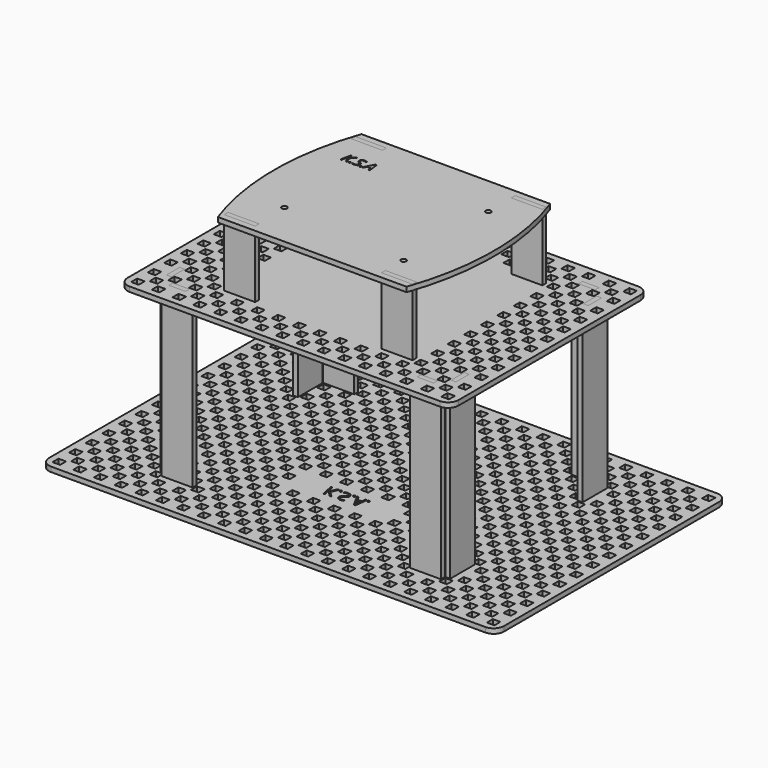
from build123d import *

# Parameters (mm, degrees)
F0_W          = 3.81
F0_H          = 3.81
F0_W_2        = 10.16
F0_H_2        = 3
F1_DEPTH      = 3
F2_W          = 10.16
F2_H          = 3
F2_W_2        = 2.9792766573
F2_W_3        = 5.9107233427
F3_DEPTH      = 3
F2_W_4        = 4.445
F4_DEPTH      = 38.1
F5_W          = 10.16
F5_H          = 3
F6_DEPTH      = 3
F7_W          = 10.16
F7_H          = 3
F7_W_2        = 3
F7_H_2        = 10.16
F8_DEPTH      = 3
F9_W          = 4.6228
F9_H          = 4.6228
F10_DEPTH     = 25.4
F11_W         = 10.16
F11_H         = 3
F12_DEPTH     = 3
F11_W_2       = 3
F11_H_2       = 10.16
F13_W         = 19.05
F13_H         = 3
F14_DEPTH     = 101.6
F13_W_2       = 3
F13_H_2       = 19.05
F15_W         = 10.16
F15_H         = 3
F16_DEPTH     = 3
F15_W_2       = 3
F15_H_2       = 10.16
F17_W         = 10.16
F17_H         = 3
F17_W_2       = 3
F17_H_2       = 10.16
F18_DEPTH     = 3
F19_W         = 4.6228
F19_H         = 4.6228
F19_TEXT_SIZE = 10.9144621995
F20_DEPTH     = 3


# Not quite as in the source:
# - Text() gives the source's letters only with a copy of the font that has no kerning and outlines rounded to 1/6400 em; it was checked with that copy


with BuildPart() as f1:
    # F0 (on Top) → F1 (new body)
    with BuildSketch(Plane.XY):
        with Locations((-97.3891888094, 47.6037588251)):
            Rectangle(F0_W, F0_H)
        with BuildLine():
            Line((-99.2941888094, 45.6987588251), (-99.2941888094, 49.5087588251))
            ThreePointArc((-99.2941888094, 49.5087588251), (-108.7600023335, -5.5912411749), (-99.2941888094, -60.6912411749))
            Line((-99.2941888094, -60.6912411749), (-99.2941888094, -56.8812411749))
            Line((-99.2941888094, -56.8812411749), (-99.2941888094, 45.6987588251))
        make_face()
        Polygon((12.7958111906, 49.5087588251), (-95.4841888094, 49.5087588251), (-95.4841888094, 45.6987588251), (-99.2941888094, 45.6987588251), (-99.2941888094, -56.8812411749), (-95.4841888094, -56.8812411749), (-95.4841888094, -60.6912411749), (12.7958111906, -60.6912411749), (12.7958111906, -56.8812411749), (16.6058111906, -56.8812411749), (16.6058111906, 42.6987588251), (12.7958111906, 42.6987588251), (2.6358111906, 42.6987588251), (2.6358111906, 45.6987588251), (12.7958111906, 45.6987588251), align=None)
        with Locations((-90.4041888094, -55.3812411749)):
            Rectangle(F0_W_2, F0_H_2, mode=Mode.SUBTRACT)
        with BuildLine():
            ThreePointArc((-80.5061888094, -34.6407411749), (-82.0936888094, -33.0532411749), (-80.5061888094, -31.4657411749))
            ThreePointArc((-80.5061888094, -31.4657411749), (-79.3836567943, -31.9307091598), (-78.9186888094, -33.0532411749))
            ThreePointArc((-78.9186888094, -33.0532411749), (-79.3836567943, -34.1757731901), (-80.5061888094, -34.6407411749))
        make_face(mode=Mode.SUBTRACT)
        with Locations((7.7158111906, -55.3812411749)):
            Rectangle(F0_W_2, F0_H_2, mode=Mode.SUBTRACT)
        with BuildLine():
            ThreePointArc((-3.1356888094, -40.2362411749), (-2.6707208245, -39.1137091598), (-1.5481888094, -38.6487411749))
            ThreePointArc((-1.5481888094, -38.6487411749), (-0.4256567943, -39.1137091598), (0.0393111906, -40.2362411749))
            ThreePointArc((0.0393111906, -40.2362411749), (-0.4256567943, -41.3587731901), (-1.5481888094, -41.8237411749))
            ThreePointArc((-1.5481888094, -41.8237411749), (-2.6707208245, -41.3587731901), (-3.1356888094, -40.2362411749))
        make_face(mode=Mode.SUBTRACT)
        with BuildLine():
            add(Edge.make_bspline(
                [(-85.8932765777, 22.6364073966), (-86.0109293332, 22.7498831312), (-86.0109293332, 22.971265239)],
                knots=[0, 0, 0, 1, 1, 1], degree=2))
            add(Edge.make_bspline(
                [(-86.0109293332, 22.971265239), (-86.0109293332, 23.3068192516), (-85.8341021149, 23.5045315744)],
                knots=[0, 0, 0, 1, 1, 1], degree=2))
            add(Edge.make_bspline(
                [(-85.8341021149, 23.5045315744), (-85.6572748967, 23.7022438971), (-85.3495676901, 23.7022438971)],
                knots=[0, 0, 0, 1, 1, 1], degree=2))
            add(Edge.make_bspline(
                [(-85.3495676901, 23.7022438971), (-85.1616017495, 23.7022438971), (-85.0467336746, 23.5894643327)],
                knots=[0, 0, 0, 1, 1, 1], degree=2))
            add(Edge.make_bspline(
                [(-85.0467336746, 23.5894643327), (-84.9318655998, 23.4766847684), (-84.9318655998, 23.2455562784)],
                knots=[0, 0, 0, 1, 1, 1], degree=2))
            add(Edge.make_bspline(
                [(-84.9318655998, 23.2455562784), (-84.9318655998, 22.9364567315), (-85.1059081374, 22.7296941968)],
                knots=[0, 0, 0, 1, 1, 1], degree=2))
            add(Edge.make_bspline(
                [(-85.1059081374, 22.7296941968), (-85.2799506751, 22.5229316621), (-85.5751268189, 22.5229316621)],
                knots=[0, 0, 0, 1, 1, 1], degree=2))
            add(Edge.make_bspline(
                [(-85.5751268189, 22.5229316621), (-85.7756238223, 22.5229316621), (-85.8932765777, 22.6364073966)],
                knots=[0, 0, 0, 1, 1, 1], degree=2))
        make_face(mode=Mode.SUBTRACT)
        with BuildLine():
            Line((-89.3609000977, 25.9216343371), (-86.5941888094, 28.7288279122))
            Line((-86.5941888094, 28.7288279122), (-86.3158518591, 29.0112374653))
            Line((-86.3158518591, 29.0112374653), (-85.4066536425, 29.0112374653))
            Line((-85.4066536425, 29.0112374653), (-86.5941888094, 27.8266770859))
            Line((-86.5941888094, 27.8266770859), (-88.1857648835, 26.2390879258))
            Line((-88.1857648835, 26.2390879258), (-86.6639369344, 22.6496346295))
            Line((-86.6639369344, 22.6496346295), (-87.4728866493, 22.6496346295))
            add(Edge.make_bspline(
                [(-87.4728866493, 22.6496346295), (-87.7861632171, 23.4376992399), (-88.1105785073, 24.2139289578)],
                knots=[0, 0, 0, 1, 1, 1], degree=2))
            add(Edge.make_bspline(
                [(-88.1105785073, 24.2139289578), (-88.4349937974, 24.9901586757), (-88.7482703652, 25.7865773279)],
                knots=[0, 0, 0, 1, 1, 1], degree=2))
            Line((-88.7482703652, 25.7865773279), (-89.5043111487, 25.2171101448))
            Line((-89.5043111487, 25.2171101448), (-90.0487162064, 22.6496346295))
            Line((-90.0487162064, 22.6496346295), (-90.7880489063, 22.6496346295))
            Line((-90.7880489063, 22.6496346295), (-89.4444405157, 29.0112374653))
            Line((-89.4444405157, 29.0112374653), (-88.7037154755, 29.0112374653))
            Line((-88.7037154755, 29.0112374653), (-89.3609000977, 25.9216343371))
        make_face(mode=Mode.SUBTRACT)
        with BuildLine():
            add(Edge.make_bspline(
                [(-79.1654882427, 22.6364073966), (-79.2831409981, 22.7498831312), (-79.2831409981, 22.971265239)],
                knots=[0, 0, 0, 1, 1, 1], degree=2))
            add(Edge.make_bspline(
                [(-79.2831409981, 22.971265239), (-79.2831409981, 23.3068192516), (-79.1063137799, 23.5045315744)],
                knots=[0, 0, 0, 1, 1, 1], degree=2))
            add(Edge.make_bspline(
                [(-79.1063137799, 23.5045315744), (-78.9294865616, 23.7022438971), (-78.6217793551, 23.7022438971)],
                knots=[0, 0, 0, 1, 1, 1], degree=2))
            add(Edge.make_bspline(
                [(-78.6217793551, 23.7022438971), (-78.4338134144, 23.7022438971), (-78.3189453396, 23.5894643327)],
                knots=[0, 0, 0, 1, 1, 1], degree=2))
            add(Edge.make_bspline(
                [(-78.3189453396, 23.5894643327), (-78.2040772648, 23.4766847684), (-78.2040772648, 23.2455562784)],
                knots=[0, 0, 0, 1, 1, 1], degree=2))
            add(Edge.make_bspline(
                [(-78.2040772648, 23.2455562784), (-78.2040772648, 22.9364567315), (-78.3781198024, 22.7296941968)],
                knots=[0, 0, 0, 1, 1, 1], degree=2))
            add(Edge.make_bspline(
                [(-78.3781198024, 22.7296941968), (-78.55216234, 22.5229316621), (-78.8473384839, 22.5229316621)],
                knots=[0, 0, 0, 1, 1, 1], degree=2))
            add(Edge.make_bspline(
                [(-78.8473384839, 22.5229316621), (-79.0478354872, 22.5229316621), (-79.1654882427, 22.6364073966)],
                knots=[0, 0, 0, 1, 1, 1], degree=2))
        make_face(mode=Mode.SUBTRACT)
        with BuildLine():
            add(Edge.make_bspline(
                [(-80.0858251817, 25.1057229207), (-80.0177086097, 24.9496740466), (-79.9899850484, 24.7637588251)],
                knots=[0, 0, 0, 0.5929982907, 0.5929982907, 0.5929982907], degree=2))
            add(Edge.make_bspline(
                [(-79.9899850484, 24.7637588251), (-79.9709571069, 24.6361567491), (-79.9709571069, 24.4944855285)],
                knots=[0.5929982907, 0.5929982907, 0.5929982907, 1, 1, 1], degree=2))
            add(Edge.make_bspline(
                [(-79.9709571069, 24.4944855285), (-79.9709571069, 23.6358738997), (-80.5061888094, 23.1363186181)],
                knots=[0, 0, 0, 0.9357631904, 0.9357631904, 0.9357631904], degree=2))
            add(Edge.make_bspline(
                [(-80.5061888094, 23.1363186181), (-80.5429305591, 23.1020259276), (-80.5821944991, 23.0694252303)],
                knots=[0.9357631904, 0.9357631904, 0.9357631904, 1, 1, 1], degree=2))
            add(Edge.make_bspline(
                [(-80.5821944991, 23.0694252303), (-81.1934318913, 22.5619171905), (-82.3031271113, 22.5619171905)],
                knots=[0, 0, 0, 1, 1, 1], degree=2))
            add(Edge.make_bspline(
                [(-82.3031271113, 22.5619171905), (-82.7639917509, 22.5619171905), (-83.1141653367, 22.6252686742)],
                knots=[0, 0, 0, 1, 1, 1], degree=2))
            add(Edge.make_bspline(
                [(-83.1141653367, 22.6252686742), (-83.4643389224, 22.6886201579), (-83.7734384693, 22.8362082298)],
                knots=[0, 0, 0, 1, 1, 1], degree=2))
            Line((-83.7734384693, 22.8362082298), (-83.7734384693, 23.57693327))
            add(Edge.make_bspline(
                [(-83.7734384693, 23.57693327), (-83.0689142769, 23.2107477708), (-82.2947730695, 23.2107477708)],
                knots=[0, 0, 0, 1, 1, 1], degree=2))
            add(Edge.make_bspline(
                [(-82.2947730695, 23.2107477708), (-81.5888565368, 23.2107477708), (-81.1760276375, 23.5393400819)],
                knots=[0, 0, 0, 1, 1, 1], degree=2))
            add(Edge.make_bspline(
                [(-81.1760276375, 23.5393400819), (-80.7631987382, 23.867932393), (-80.7631987382, 24.4429689373)],
                knots=[0, 0, 0, 1, 1, 1], degree=2))
            add(Edge.make_bspline(
                [(-80.7631987382, 24.4429689373), (-80.7631987382, 24.7813076305), (-80.9915425476, 25.0402829265)],
                knots=[0, 0, 0, 1, 1, 1], degree=2))
            add(Edge.make_bspline(
                [(-80.9915425476, 25.0402829265), (-81.219886357, 25.2992582225), (-81.8422624716, 25.6515203187)],
                knots=[0, 0, 0, 1, 1, 1], degree=2))
            add(Edge.make_bspline(
                [(-81.8422624716, 25.6515203187), (-82.4980547534, 26.0218828388), (-82.7528530285, 26.3915491888)],
                knots=[0, 0, 0, 1, 1, 1], degree=2))
            add(Edge.make_bspline(
                [(-82.7528530285, 26.3915491888), (-83.0076513036, 26.7612155387), (-83.0076513036, 27.266635068)],
                knots=[0, 0, 0, 1, 1, 1], degree=2))
            add(Edge.make_bspline(
                [(-83.0076513036, 27.266635068), (-83.0076513036, 28.0797618039), (-82.4333109294, 28.5907506944)],
                knots=[0, 0, 0, 1, 1, 1], degree=2))
            add(Edge.make_bspline(
                [(-82.4333109294, 28.5907506944), (-81.8589705552, 29.1017395849), (-80.9233178729, 29.1017395849)],
                knots=[0, 0, 0, 1, 1, 1], degree=2))
            add(Edge.make_bspline(
                [(-80.9233178729, 29.1017395849), (-80.4930847198, 29.1017395849), (-80.1206336893, 29.0195915071)],
                knots=[0, 0, 0, 1, 1, 1], degree=2))
            add(Edge.make_bspline(
                [(-80.1206336893, 29.0195915071), (-79.7481826587, 28.9374434294), (-79.3360499296, 28.736946426)],
                knots=[0, 0, 0, 1, 1, 1], degree=2))
            Line((-79.3360499296, 28.736946426), (-79.6228720316, 28.0839388248))
            add(Edge.make_bspline(
                [(-79.6228720316, 28.0839388248), (-79.9096941336, 28.2496273206), (-80.2668294209, 28.3450026312)],
                knots=[0, 0, 0, 1, 1, 1], degree=2))
            add(Edge.make_bspline(
                [(-80.2668294209, 28.3450026312), (-80.6239647081, 28.4403779419), (-80.9233178729, 28.4403779419)],
                knots=[0, 0, 0, 1, 1, 1], degree=2))
            add(Edge.make_bspline(
                [(-80.9233178729, 28.4403779419), (-81.506708459, 28.4403779419), (-81.8610590657, 28.1382400965)],
                knots=[0, 0, 0, 1, 1, 1], degree=2))
            add(Edge.make_bspline(
                [(-81.8610590657, 28.1382400965), (-82.2154096723, 27.8361022512), (-82.2154096723, 27.3181516592)],
                knots=[0, 0, 0, 1, 1, 1], degree=2))
            add(Edge.make_bspline(
                [(-82.2154096723, 27.3181516592), (-82.2154096723, 27.0828461483), (-82.1416156363, 26.9157653121)],
                knots=[0, 0, 0, 1, 1, 1], degree=2))
            add(Edge.make_bspline(
                [(-82.1416156363, 26.9157653121), (-82.0678216004, 26.748684476), (-81.9070062956, 26.6004002339)],
                knots=[0, 0, 0, 1, 1, 1], degree=2))
            add(Edge.make_bspline(
                [(-81.9070062956, 26.6004002339), (-81.7461909908, 26.4521159919), (-81.2895033721, 26.1875713346)],
                knots=[0, 0, 0, 1, 1, 1], degree=2))
            add(Edge.make_bspline(
                [(-81.2895033721, 26.1875713346), (-80.6490268335, 25.8046777518), (-80.4248600451, 25.5867764947)],
                knots=[0, 0, 0, 1, 1, 1], degree=2))
            add(Edge.make_bspline(
                [(-80.4248600451, 25.5867764947), (-80.2006932566, 25.3688752376), (-80.0858251817, 25.1057229207)],
                knots=[0, 0, 0, 1, 1, 1], degree=2))
        make_face(mode=Mode.SUBTRACT)
        Polygon((-73.4910053454, 29.0112374653), (-72.9564681999, 24.7637588251), (-72.6904096723, 22.6496346295), (-73.4297423722, 22.6496346295), (-73.6775789458, 24.672705087), (-75.8357064125, 24.672705087), (-76.9022390832, 22.6496346295), (-77.7251122012, 22.6496346295), (-76.5697241258, 24.7637588251), (-74.2484384693, 29.0112374653), align=None, mode=Mode.SUBTRACT)
        with Locations((-90.4041888094, 44.1987588251)):
            Rectangle(F0_W_2, F0_H_2, mode=Mode.SUBTRACT)
        with BuildLine():
            ThreePointArc((-3.1356888094, 24.7637588251), (-2.6707208245, 25.8862908402), (-1.5481888094, 26.3512588251))
            ThreePointArc((-1.5481888094, 26.3512588251), (-0.4256567943, 25.8862908402), (0.0393111906, 24.7637588251))
            ThreePointArc((0.0393111906, 24.7637588251), (-0.4256567943, 23.6412268099), (-1.5481888094, 23.1762588251))
            ThreePointArc((-1.5481888094, 23.1762588251), (-2.6707208245, 23.6412268099), (-3.1356888094, 24.7637588251))
        make_face(mode=Mode.SUBTRACT)
        with Locations((-97.3891888094, -58.7862411749)):
            Rectangle(F0_W, F0_H)
        Polygon((16.6058111906, 49.5087588251), (12.7958111906, 49.5087588251), (12.7958111906, 45.6987588251), (12.7958111906, 42.6987588251), (16.6058111906, 42.6987588251), align=None)
        with BuildLine():
            ThreePointArc((16.6058111906, -60.6912411749), (26.0716247148, -5.5912411749), (16.6058111906, 49.5087588251))
            Line((16.6058111906, 49.5087588251), (16.6058111906, 42.6987588251))
            Line((16.6058111906, 42.6987588251), (16.6058111906, -56.8812411749))
            Line((16.6058111906, -56.8812411749), (16.6058111906, -60.6912411749))
        make_face()
        with Locations((14.7008111906, -58.7862411749)):
            Rectangle(F0_W, F0_H)
    extrude(amount=F1_DEPTH)


with BuildPart() as f3:
    # F2 (on face) → F3 (new body)
    with BuildSketch(Plane(origin=(0, 0, 0), x_dir=(1, 0, 0), z_dir=(0, 0, -1))):
        with Locations((-90.4041888094, 55.3812411749)):
            Rectangle(F2_W, F2_H)
        with Locations((-96.9738271381, 55.3812411749)):
            Rectangle(F2_W_2, F2_H)
        with Locations((-82.3688271381, 55.3812411749)):
            Rectangle(F2_W_3, F2_H)
    extrude(amount=-F3_DEPTH)

    # F4 (add): a face of the model
    f4_faces = [f3.faces().sort_by_distance(p)[0] for p in [
        (-88.9384654667, -55.3812411749, 0),
    ]]
    extrude(f4_faces, amount=F4_DEPTH)

    # F5 (on face) → F6 (join)
    with BuildSketch(Plane(origin=(0, 0, -38.1), x_dir=(1, 0, 0), z_dir=(0, 0, -1))):
        with Locations((-88.9384654667, 55.3812411749)):
            Rectangle(F5_W, F5_H)
    extrude(amount=F6_DEPTH)


with BuildPart() as f3b:
    # F2 (on face) → F3, piece 2 (new body)
    with BuildSketch(Plane(origin=(0, 0, 0), x_dir=(1, 0, 0), z_dir=(0, 0, -1))):
        with Locations((7.7158111906, 55.3812411749)):
            Rectangle(F2_W, F2_H)
        with Locations((0.4133111906, 55.3812411749)):
            Rectangle(F2_W_4, F2_H)
        with Locations((15.0183111906, 55.3812411749)):
            Rectangle(F2_W_4, F2_H)
    extrude(amount=-F3_DEPTH)

    # F4#2 (add): a face of the model
    f4_2_faces = [f3b.faces().sort_by_distance(p)[0] for p in [
        (7.7158111906, -55.3812411749, 0),
    ]]
    extrude(f4_2_faces, amount=F4_DEPTH)

    # F5 (on face) → F6, piece 2 (join)
    with BuildSketch(Plane(origin=(0, 0, -38.1), x_dir=(1, 0, 0), z_dir=(0, 0, -1))):
        with Locations((7.7158111906, 55.3812411749)):
            Rectangle(F5_W, F5_H)
    extrude(amount=F6_DEPTH)


with BuildPart() as f3c:
    # F2 (on face) → F3, piece 3 (new body)
    with BuildSketch(Plane(origin=(0, 0, 0), x_dir=(1, 0, 0), z_dir=(0, 0, -1))):
        with Locations((-90.4041888094, -44.1987588251)):
            Rectangle(F2_W, F2_H)
        with Locations((-97.7066888094, -44.1987588251)):
            Rectangle(F2_W_4, F2_H)
        with Locations((-83.1016888094, -44.1987588251)):
            Rectangle(F2_W_4, F2_H)
    extrude(amount=-F3_DEPTH)

    # F4#3 (add): a face of the model
    f4_3_faces = [f3c.faces().sort_by_distance(p)[0] for p in [
        (-90.4041888094, 44.1987588251, 0),
    ]]
    extrude(f4_3_faces, amount=F4_DEPTH)

    # F5 (on face) → F6, piece 4 (join)
    with BuildSketch(Plane(origin=(0, 0, -38.1), x_dir=(1, 0, 0), z_dir=(0, 0, -1))):
        with Locations((-90.4041888094, -44.1987588251)):
            Rectangle(F5_W, F5_H)
    extrude(amount=F6_DEPTH)


with BuildPart() as f3d:
    # F2 (on face) → F3, piece 4 (new body)
    with BuildSketch(Plane(origin=(0, 0, 0), x_dir=(1, 0, 0), z_dir=(0, 0, -1))):
        with Locations((7.7158111906, -44.1987588251)):
            Rectangle(F2_W, F2_H)
        with Locations((0.4133111906, -44.1987588251)):
            Rectangle(F2_W_4, F2_H)
        with Locations((15.0183111906, -44.1987588251)):
            Rectangle(F2_W_4, F2_H)
    extrude(amount=-F3_DEPTH)

    # F4#4 (add): a face of the model
    f4_4_faces = [f3d.faces().sort_by_distance(p)[0] for p in [
        (7.7158111906, 44.1987588251, 0),
    ]]
    extrude(f4_4_faces, amount=F4_DEPTH)

    # F5 (on face) → F6, piece 3 (join)
    with BuildSketch(Plane(origin=(0, 0, -38.1), x_dir=(1, 0, 0), z_dir=(0, 0, -1))):
        with Locations((7.7158111906, -44.1987588251)):
            Rectangle(F5_W, F5_H)
    extrude(amount=F6_DEPTH)


with BuildPart() as f8:
    # F7 (on face) → F8 (new body)
    with BuildSketch(Plane(origin=(0, 0, -41.1), x_dir=(1, 0, 0), z_dir=(0, 0, -1))):
        with BuildLine():
            Line((-41.3441888094, 81.7912411749), (-136.5941888094, 81.7912411749))
            ThreePointArc((-136.5941888094, 81.7912411749), (-141.0843168699, 79.9313692355), (-142.9441888094, 75.4412411749))
            Line((-142.9441888094, 75.4412411749), (-142.9441888094, -64.2587588251))
            ThreePointArc((-142.9441888094, -64.2587588251), (-141.0843168699, -68.7488868856), (-136.5941888094, -70.6087588251))
            Line((-136.5941888094, -70.6087588251), (-41.3441888094, -70.6087588251))
            Line((-41.3441888094, -70.6087588251), (53.9058111906, -70.6087588251))
            ThreePointArc((53.9058111906, -70.6087588251), (58.3959392511, -68.7488868856), (60.2558111906, -64.2587588251))
            Line((60.2558111906, -64.2587588251), (60.2558111906, 75.4412411749))
            ThreePointArc((60.2558111906, 75.4412411749), (58.3959392511, 79.9313692355), (53.9058111906, 81.7912411749))
            Line((53.9058111906, 81.7912411749), (-41.3441888094, 81.7912411749))
        make_face()
        with Locations((-117.5441888094, -56.4087588251)):
            Rectangle(F7_W, F7_H, mode=Mode.SUBTRACT)
        with Locations((-128.7441888094, -45.2087588251)):
            Rectangle(F7_W_2, F7_H_2, mode=Mode.SUBTRACT)
        with Locations((-90.4041888094, -44.1987588251)):
            Rectangle(F7_W, F7_H, mode=Mode.SUBTRACT)
        with Locations((7.7158111906, -44.1987588251)):
            Rectangle(F7_W, F7_H, mode=Mode.SUBTRACT)
        with Locations((34.8558111906, -56.4087588251)):
            Rectangle(F7_W, F7_H, mode=Mode.SUBTRACT)
        with Locations((46.0558111906, -45.2087588251)):
            Rectangle(F7_W_2, F7_H_2, mode=Mode.SUBTRACT)
        with Locations((-128.7441888094, 56.3912411749)):
            Rectangle(F7_W_2, F7_H_2, mode=Mode.SUBTRACT)
        with Locations((-117.5441888094, 67.5912411749)):
            Rectangle(F7_W, F7_H, mode=Mode.SUBTRACT)
        with Locations((-88.9384654667, 55.3812411749)):
            Rectangle(F7_W, F7_H, mode=Mode.SUBTRACT)
        with Locations((7.7158111906, 55.3812411749)):
            Rectangle(F7_W, F7_H, mode=Mode.SUBTRACT)
        with Locations((46.0558111906, 56.3912411749)):
            Rectangle(F7_W_2, F7_H_2, mode=Mode.SUBTRACT)
        with Locations((34.8558111906, 67.5912411749)):
            Rectangle(F7_W, F7_H, mode=Mode.SUBTRACT)
    extrude(amount=-F8_DEPTH)

    # F9 (on face) → F10 (cut)
    with BuildSketch(Plane(origin=(0, 0, -41.1), x_dir=(1, 0, 0), z_dir=(0, 0, -1))):
        with Locations((-123.8941888094, 75.4412411749)):
            Rectangle(F9_W, F9_H)
        with Locations((-136.5941888094, 62.7412411749)):
            Rectangle(F9_W, F9_H)
        with Locations((-130.2441888094, 69.0912411749)):
            Rectangle(F9_W, F9_H)
        Polygon((-136.5941888094, 77.7526411749), (-138.9055888094, 77.7526411749), (-138.9055888094, 75.4412411749), (-138.9055888094, 73.1298411749), (-134.2827888094, 73.1298411749), (-134.2827888094, 77.7526411749), align=None)
        with Locations((-136.5941888094, 50.0412411749)):
            Rectangle(F9_W, F9_H)
        with Locations((-136.5941888094, 37.3412411749)):
            Rectangle(F9_W, F9_H)
        with Locations((-136.5941888094, 24.6412411749)):
            Rectangle(F9_W, F9_H)
        with Locations((-136.5941888094, 11.9412411749)):
            Rectangle(F9_W, F9_H)
        with Locations((-136.5941888094, -0.7587588251)):
            Rectangle(F9_W, F9_H)
        with Locations((-136.5941888094, -13.4587588251)):
            Rectangle(F9_W, F9_H)
        with Locations((-136.5941888094, -26.1587588251)):
            Rectangle(F9_W, F9_H)
        with Locations((-136.5941888094, -38.8587588251)):
            Rectangle(F9_W, F9_H)
        with Locations((-136.5941888094, -51.5587588251)):
            Rectangle(F9_W, F9_H)
        Polygon((-134.2827888094, -66.5701588251), (-134.2827888094, -61.9473588251), (-138.9055888094, -61.9473588251), (-138.9055888094, -66.5701588251), (-136.5941888094, -66.5701588251), align=None)
        with Locations((-123.8941888094, 62.7412411749)):
            Rectangle(F9_W, F9_H)
        with Locations((-123.8941888094, 50.0412411749)):
            Rectangle(F9_W, F9_H)
        with Locations((-123.8941888094, 37.3412411749)):
            Rectangle(F9_W, F9_H)
        with Locations((-123.8941888094, 24.6412411749)):
            Rectangle(F9_W, F9_H)
        with Locations((-123.8941888094, 11.9412411749)):
            Rectangle(F9_W, F9_H)
        with Locations((-123.8941888094, -0.7587588251)):
            Rectangle(F9_W, F9_H)
        with Locations((-123.8941888094, -13.4587588251)):
            Rectangle(F9_W, F9_H)
        with Locations((-123.8941888094, -26.1587588251)):
            Rectangle(F9_W, F9_H)
        with Locations((-123.8941888094, -38.8587588251)):
            Rectangle(F9_W, F9_H)
        with Locations((-123.8941888094, -51.5587588251)):
            Rectangle(F9_W, F9_H)
        with Locations((-123.8941888094, -64.2587588251)):
            Rectangle(F9_W, F9_H)
        with Locations((-111.1941888094, 75.4412411749)):
            Rectangle(F9_W, F9_H)
        with Locations((-111.1941888094, 62.7412411749)):
            Rectangle(F9_W, F9_H)
        with Locations((-111.1941888094, 50.0412411749)):
            Rectangle(F9_W, F9_H)
        with Locations((-111.1941888094, 37.3412411749)):
            Rectangle(F9_W, F9_H)
        with Locations((-111.1941888094, 24.6412411749)):
            Rectangle(F9_W, F9_H)
        with Locations((-111.1941888094, 11.9412411749)):
            Rectangle(F9_W, F9_H)
        with Locations((-111.1941888094, -0.7587588251)):
            Rectangle(F9_W, F9_H)
        with Locations((-111.1941888094, -13.4587588251)):
            Rectangle(F9_W, F9_H)
        with Locations((-111.1941888094, -26.1587588251)):
            Rectangle(F9_W, F9_H)
        with Locations((-111.1941888094, -38.8587588251)):
            Rectangle(F9_W, F9_H)
        with Locations((-111.1941888094, -51.5587588251)):
            Rectangle(F9_W, F9_H)
        with Locations((-111.1941888094, -64.2587588251)):
            Rectangle(F9_W, F9_H)
        with Locations((-98.4941888094, 75.4412411749)):
            Rectangle(F9_W, F9_H)
        with Locations((-98.4941888094, 62.7412411749)):
            Rectangle(F9_W, F9_H)
        with Locations((-98.4941888094, -51.5587588251)):
            Rectangle(F9_W, F9_H)
        with Locations((-98.4941888094, -64.2587588251)):
            Rectangle(F9_W, F9_H)
        with Locations((-85.7941888094, 75.4412411749)):
            Rectangle(F9_W, F9_H)
        with Locations((-85.7941888094, 62.7412411749)):
            Rectangle(F9_W, F9_H)
        with Locations((-85.7941888094, -51.5587588251)):
            Rectangle(F9_W, F9_H)
        with Locations((-85.7941888094, -64.2587588251)):
            Rectangle(F9_W, F9_H)
        with Locations((-73.0941888094, 75.4412411749)):
            Rectangle(F9_W, F9_H)
        with Locations((-73.0941888094, 62.7412411749)):
            Rectangle(F9_W, F9_H)
        with Locations((-73.0941888094, -51.5587588251)):
            Rectangle(F9_W, F9_H)
        with Locations((-73.0941888094, -64.2587588251)):
            Rectangle(F9_W, F9_H)
        with Locations((-60.3941888094, 75.4412411749)):
            Rectangle(F9_W, F9_H)
        with Locations((-60.3941888094, 62.7412411749)):
            Rectangle(F9_W, F9_H)
        with Locations((-60.3941888094, -51.5587588251)):
            Rectangle(F9_W, F9_H)
        with Locations((-60.3941888094, -64.2587588251)):
            Rectangle(F9_W, F9_H)
        with Locations((-47.6941888094, 75.4412411749)):
            Rectangle(F9_W, F9_H)
        with Locations((-47.6941888094, 62.7412411749)):
            Rectangle(F9_W, F9_H)
        with Locations((-47.6941888094, -51.5587588251)):
            Rectangle(F9_W, F9_H)
        with Locations((-47.6941888094, -64.2587588251)):
            Rectangle(F9_W, F9_H)
        with Locations((-34.9941888094, 75.4412411749)):
            Rectangle(F9_W, F9_H)
        with Locations((-34.9941888094, 62.7412411749)):
            Rectangle(F9_W, F9_H)
        with Locations((-34.9941888094, -51.5587588251)):
            Rectangle(F9_W, F9_H)
        with Locations((-34.9941888094, -64.2587588251)):
            Rectangle(F9_W, F9_H)
        with Locations((-22.2941888094, 75.4412411749)):
            Rectangle(F9_W, F9_H)
        with Locations((-22.2941888094, 62.7412411749)):
            Rectangle(F9_W, F9_H)
        with Locations((-22.2941888094, -51.5587588251)):
            Rectangle(F9_W, F9_H)
        with Locations((-22.2941888094, -64.2587588251)):
            Rectangle(F9_W, F9_H)
        with Locations((-9.5941888094, 75.4412411749)):
            Rectangle(F9_W, F9_H)
        with Locations((-9.5941888094, 62.7412411749)):
            Rectangle(F9_W, F9_H)
        with Locations((-9.5941888094, -51.5587588251)):
            Rectangle(F9_W, F9_H)
        with Locations((-9.5941888094, -64.2587588251)):
            Rectangle(F9_W, F9_H)
        with Locations((3.1058111906, 75.4412411749)):
            Rectangle(F9_W, F9_H)
        with Locations((3.1058111906, 62.7412411749)):
            Rectangle(F9_W, F9_H)
        with Locations((3.1058111906, -51.5587588251)):
            Rectangle(F9_W, F9_H)
        with Locations((3.1058111906, -64.2587588251)):
            Rectangle(F9_W, F9_H)
        with Locations((15.8058111906, 75.4412411749)):
            Rectangle(F9_W, F9_H)
        with Locations((15.8058111906, 62.7412411749)):
            Rectangle(F9_W, F9_H)
        with Locations((15.8058111906, -51.5587588251)):
            Rectangle(F9_W, F9_H)
        with Locations((15.8058111906, -64.2587588251)):
            Rectangle(F9_W, F9_H)
        with Locations((28.5058111906, 75.4412411749)):
            Rectangle(F9_W, F9_H)
        with Locations((28.5058111906, 62.7412411749)):
            Rectangle(F9_W, F9_H)
        with Locations((28.5058111906, 50.0412411749)):
            Rectangle(F9_W, F9_H)
        with Locations((28.5058111906, 37.3412411749)):
            Rectangle(F9_W, F9_H)
        with Locations((28.5058111906, 24.6412411749)):
            Rectangle(F9_W, F9_H)
        with Locations((28.5058111906, 11.9412411749)):
            Rectangle(F9_W, F9_H)
        with Locations((28.5058111906, -0.7587588251)):
            Rectangle(F9_W, F9_H)
        with Locations((28.5058111906, -13.4587588251)):
            Rectangle(F9_W, F9_H)
        with Locations((28.5058111906, -26.1587588251)):
            Rectangle(F9_W, F9_H)
        with Locations((28.5058111906, -38.8587588251)):
            Rectangle(F9_W, F9_H)
        with Locations((28.5058111906, -51.5587588251)):
            Rectangle(F9_W, F9_H)
        with Locations((28.5058111906, -64.2587588251)):
            Rectangle(F9_W, F9_H)
        with Locations((41.2058111906, 75.4412411749)):
            Rectangle(F9_W, F9_H)
        with Locations((41.2058111906, 62.7412411749)):
            Rectangle(F9_W, F9_H)
        with Locations((41.2058111906, 50.0412411749)):
            Rectangle(F9_W, F9_H)
        with Locations((41.2058111906, 37.3412411749)):
            Rectangle(F9_W, F9_H)
        with Locations((41.2058111906, 24.6412411749)):
            Rectangle(F9_W, F9_H)
        with Locations((41.2058111906, 11.9412411749)):
            Rectangle(F9_W, F9_H)
        with Locations((41.2058111906, -0.7587588251)):
            Rectangle(F9_W, F9_H)
        with Locations((41.2058111906, -13.4587588251)):
            Rectangle(F9_W, F9_H)
        with Locations((41.2058111906, -26.1587588251)):
            Rectangle(F9_W, F9_H)
        with Locations((41.2058111906, -38.8587588251)):
            Rectangle(F9_W, F9_H)
        with Locations((41.2058111906, -51.5587588251)):
            Rectangle(F9_W, F9_H)
        with Locations((41.2058111906, -64.2587588251)):
            Rectangle(F9_W, F9_H)
        Polygon((56.2172111906, 75.4412411749), (56.2172111906, 77.7526411749), (51.5944111906, 77.7526411749), (51.5944111906, 73.1298411749), (56.2172111906, 73.1298411749), align=None)
        with Locations((53.9058111906, 62.7412411749)):
            Rectangle(F9_W, F9_H)
        with Locations((53.9058111906, 50.0412411749)):
            Rectangle(F9_W, F9_H)
        with Locations((53.9058111906, 37.3412411749)):
            Rectangle(F9_W, F9_H)
        with Locations((53.9058111906, 24.6412411749)):
            Rectangle(F9_W, F9_H)
        with Locations((53.9058111906, 11.9412411749)):
            Rectangle(F9_W, F9_H)
        with Locations((53.9058111906, -0.7587588251)):
            Rectangle(F9_W, F9_H)
        with Locations((53.9058111906, -13.4587588251)):
            Rectangle(F9_W, F9_H)
        with Locations((53.9058111906, -26.1587588251)):
            Rectangle(F9_W, F9_H)
        with Locations((53.9058111906, -38.8587588251)):
            Rectangle(F9_W, F9_H)
        with Locations((53.9058111906, -51.5587588251)):
            Rectangle(F9_W, F9_H)
        with Locations((53.9058111906, -64.2587588251)):
            Rectangle(F9_W, F9_H)
        with Locations((-130.2441888094, 43.6912411749)):
            Rectangle(F9_W, F9_H)
        with Locations((-130.2441888094, 30.9912411749)):
            Rectangle(F9_W, F9_H)
        with Locations((-130.2441888094, 18.2912411749)):
            Rectangle(F9_W, F9_H)
        with Locations((-130.2441888094, 5.5912411749)):
            Rectangle(F9_W, F9_H)
        with Locations((-130.2441888094, -7.1087588251)):
            Rectangle(F9_W, F9_H)
        with Locations((-130.2441888094, -19.8087588251)):
            Rectangle(F9_W, F9_H)
        with Locations((-130.2441888094, -32.5087588251)):
            Rectangle(F9_W, F9_H)
        with Locations((-130.2441888094, -57.9087588251)):
            Rectangle(F9_W, F9_H)
        with Locations((-117.5441888094, 56.3912411749)):
            Rectangle(F9_W, F9_H)
        with Locations((-117.5441888094, 43.6912411749)):
            Rectangle(F9_W, F9_H)
        with Locations((-117.5441888094, 30.9912411749)):
            Rectangle(F9_W, F9_H)
        with Locations((-117.5441888094, 18.2912411749)):
            Rectangle(F9_W, F9_H)
        with Locations((-117.5441888094, 5.5912411749)):
            Rectangle(F9_W, F9_H)
        with Locations((-117.5441888094, -7.1087588251)):
            Rectangle(F9_W, F9_H)
        with Locations((-117.5441888094, -19.8087588251)):
            Rectangle(F9_W, F9_H)
        with Locations((-117.5441888094, -32.5087588251)):
            Rectangle(F9_W, F9_H)
        with Locations((-117.5441888094, -45.2087588251)):
            Rectangle(F9_W, F9_H)
        with Locations((-104.8441888094, 69.0912411749)):
            Rectangle(F9_W, F9_H)
        with Locations((-104.8441888094, 56.3912411749)):
            Rectangle(F9_W, F9_H)
        with Locations((-104.8441888094, 43.6912411749)):
            Rectangle(F9_W, F9_H)
        with Locations((-104.8441888094, 30.9912411749)):
            Rectangle(F9_W, F9_H)
        with Locations((-104.8441888094, 18.2912411749)):
            Rectangle(F9_W, F9_H)
        with Locations((-104.8441888094, 5.5912411749)):
            Rectangle(F9_W, F9_H)
        with Locations((-104.8441888094, -7.1087588251)):
            Rectangle(F9_W, F9_H)
        with Locations((-104.8441888094, -19.8087588251)):
            Rectangle(F9_W, F9_H)
        with Locations((-104.8441888094, -32.5087588251)):
            Rectangle(F9_W, F9_H)
        with Locations((-104.8441888094, -45.2087588251)):
            Rectangle(F9_W, F9_H)
        with Locations((-104.8441888094, -57.9087588251)):
            Rectangle(F9_W, F9_H)
        with Locations((-92.1441888094, 69.0912411749)):
            Rectangle(F9_W, F9_H)
        with Locations((-92.1441888094, -57.9087588251)):
            Rectangle(F9_W, F9_H)
        with Locations((-79.4441888094, 69.0912411749)):
            Rectangle(F9_W, F9_H)
        with Locations((-79.4441888094, -57.9087588251)):
            Rectangle(F9_W, F9_H)
        with Locations((-66.7441888094, 69.0912411749)):
            Rectangle(F9_W, F9_H)
        with Locations((-66.7441888094, -57.9087588251)):
            Rectangle(F9_W, F9_H)
        with Locations((-54.0441888094, 69.0912411749)):
            Rectangle(F9_W, F9_H)
        with Locations((-54.0441888094, -57.9087588251)):
            Rectangle(F9_W, F9_H)
        with Locations((-41.3441888094, 69.0912411749)):
            Rectangle(F9_W, F9_H)
        with Locations((-41.3441888094, -57.9087588251)):
            Rectangle(F9_W, F9_H)
        with Locations((-28.6441888094, 69.0912411749)):
            Rectangle(F9_W, F9_H)
        with Locations((-28.6441888094, -57.9087588251)):
            Rectangle(F9_W, F9_H)
        with Locations((-15.9441888094, 69.0912411749)):
            Rectangle(F9_W, F9_H)
        with Locations((-15.9441888094, -57.9087588251)):
            Rectangle(F9_W, F9_H)
        with Locations((-3.2441888094, 69.0912411749)):
            Rectangle(F9_W, F9_H)
        with Locations((-3.2441888094, -57.9087588251)):
            Rectangle(F9_W, F9_H)
        with Locations((9.4558111906, 69.0912411749)):
            Rectangle(F9_W, F9_H)
        with Locations((9.4558111906, -57.9087588251)):
            Rectangle(F9_W, F9_H)
        with Locations((22.1558111906, 69.0912411749)):
            Rectangle(F9_W, F9_H)
        with Locations((22.1558111906, 56.3912411749)):
            Rectangle(F9_W, F9_H)
        with Locations((22.1558111906, 43.6912411749)):
            Rectangle(F9_W, F9_H)
        with Locations((22.1558111906, 30.9912411749)):
            Rectangle(F9_W, F9_H)
        with Locations((22.1558111906, 18.2912411749)):
            Rectangle(F9_W, F9_H)
        with Locations((22.1558111906, 5.5912411749)):
            Rectangle(F9_W, F9_H)
        with Locations((22.1558111906, -7.1087588251)):
            Rectangle(F9_W, F9_H)
        with Locations((22.1558111906, -19.8087588251)):
            Rectangle(F9_W, F9_H)
        with Locations((22.1558111906, -32.5087588251)):
            Rectangle(F9_W, F9_H)
        with Locations((22.1558111906, -45.2087588251)):
            Rectangle(F9_W, F9_H)
        with Locations((22.1558111906, -57.9087588251)):
            Rectangle(F9_W, F9_H)
        with Locations((34.8558111906, 56.3912411749)):
            Rectangle(F9_W, F9_H)
        with Locations((34.8558111906, 43.6912411749)):
            Rectangle(F9_W, F9_H)
        with Locations((34.8558111906, 30.9912411749)):
            Rectangle(F9_W, F9_H)
        with Locations((34.8558111906, 18.2912411749)):
            Rectangle(F9_W, F9_H)
        with Locations((34.8558111906, 5.5912411749)):
            Rectangle(F9_W, F9_H)
        with Locations((34.8558111906, -7.1087588251)):
            Rectangle(F9_W, F9_H)
        with Locations((34.8558111906, -19.8087588251)):
            Rectangle(F9_W, F9_H)
        with Locations((34.8558111906, -32.5087588251)):
            Rectangle(F9_W, F9_H)
        with Locations((34.8558111906, -45.2087588251)):
            Rectangle(F9_W, F9_H)
        with Locations((47.5558111906, 69.0912411749)):
            Rectangle(F9_W, F9_H)
        with Locations((47.5558111906, 43.6912411749)):
            Rectangle(F9_W, F9_H)
        with Locations((47.5558111906, 30.9912411749)):
            Rectangle(F9_W, F9_H)
        with Locations((47.5558111906, 18.2912411749)):
            Rectangle(F9_W, F9_H)
        with Locations((47.5558111906, 5.5912411749)):
            Rectangle(F9_W, F9_H)
        with Locations((47.5558111906, -7.1087588251)):
            Rectangle(F9_W, F9_H)
        with Locations((47.5558111906, -19.8087588251)):
            Rectangle(F9_W, F9_H)
        with Locations((47.5558111906, -32.5087588251)):
            Rectangle(F9_W, F9_H)
        with Locations((47.5558111906, -57.9087588251)):
            Rectangle(F9_W, F9_H)
    extrude(amount=-F10_DEPTH, mode=Mode.SUBTRACT)


with BuildPart() as f12:
    # F11 (on face) → F12 (new body)
    with BuildSketch(Plane(origin=(0, 0, -41.1), x_dir=(1, 0, 0), z_dir=(0, 0, -1))):
        with Locations((-117.5441888094, 67.5912411749)):
            Rectangle(F11_W, F11_H)
    extrude(amount=-F12_DEPTH)

    # F13 (on face) → F14 (join)
    with BuildSketch(Plane(origin=(0, 0, -41.1), x_dir=(1, 0, 0), z_dir=(0, 0, -1))):
        with Locations((-117.5441888094, 67.5912411749)):
            Rectangle(F13_W, F13_H)
    extrude(amount=F14_DEPTH)

    # F15 (on face) → F16 (join)
    with BuildSketch(Plane(origin=(0, 0, -142.7), x_dir=(1, 0, 0), z_dir=(0, 0, -1))):
        with Locations((-117.5441888094, 67.5912411749)):
            Rectangle(F15_W, F15_H)
    extrude(amount=F16_DEPTH)


with BuildPart() as f12b:
    # F11 (on face) → F12, piece 2 (new body)
    with BuildSketch(Plane(origin=(0, 0, -41.1), x_dir=(1, 0, 0), z_dir=(0, 0, -1))):
        with Locations((-128.7441888094, 56.3912411749)):
            Rectangle(F11_W_2, F11_H_2)
    extrude(amount=-F12_DEPTH)

    # F13 (on face) → F14, piece 2 (join)
    with BuildSketch(Plane(origin=(0, 0, -41.1), x_dir=(1, 0, 0), z_dir=(0, 0, -1))):
        with Locations((-128.7441888094, 56.3912411749)):
            Rectangle(F13_W_2, F13_H_2)
    extrude(amount=F14_DEPTH)

    # F15 (on face) → F16, piece 2 (join)
    with BuildSketch(Plane(origin=(0, 0, -142.7), x_dir=(1, 0, 0), z_dir=(0, 0, -1))):
        with Locations((-128.7441888094, 56.3912411749)):
            Rectangle(F15_W_2, F15_H_2)
    extrude(amount=F16_DEPTH)


with BuildPart() as f12c:
    # F11 (on face) → F12, piece 3 (new body)
    with BuildSketch(Plane(origin=(0, 0, -41.1), x_dir=(1, 0, 0), z_dir=(0, 0, -1))):
        with Locations((-128.7441888094, -45.2087588251)):
            Rectangle(F11_W_2, F11_H_2)
    extrude(amount=-F12_DEPTH)

    # F13 (on face) → F14, piece 6 (join)
    with BuildSketch(Plane(origin=(0, 0, -41.1), x_dir=(1, 0, 0), z_dir=(0, 0, -1))):
        with Locations((-128.7441888094, -45.2087588251)):
            Rectangle(F13_W_2, F13_H_2)
    extrude(amount=F14_DEPTH)

    # F15 (on face) → F16, piece 8 (join)
    with BuildSketch(Plane(origin=(0, 0, -142.7), x_dir=(1, 0, 0), z_dir=(0, 0, -1))):
        with Locations((-128.7441888094, -45.2087588251)):
            Rectangle(F15_W_2, F15_H_2)
    extrude(amount=F16_DEPTH)


with BuildPart() as f12d:
    # F11 (on face) → F12, piece 4 (new body)
    with BuildSketch(Plane(origin=(0, 0, -41.1), x_dir=(1, 0, 0), z_dir=(0, 0, -1))):
        with Locations((-117.5441888094, -56.4087588251)):
            Rectangle(F11_W, F11_H)
    extrude(amount=-F12_DEPTH)

    # F13 (on face) → F14, piece 7 (join)
    with BuildSketch(Plane(origin=(0, 0, -41.1), x_dir=(1, 0, 0), z_dir=(0, 0, -1))):
        with Locations((-117.5441888094, -56.4087588251)):
            Rectangle(F13_W, F13_H)
    extrude(amount=F14_DEPTH)

    # F15 (on face) → F16, piece 7 (join)
    with BuildSketch(Plane(origin=(0, 0, -142.7), x_dir=(1, 0, 0), z_dir=(0, 0, -1))):
        with Locations((-117.5441888094, -56.4087588251)):
            Rectangle(F15_W, F15_H)
    extrude(amount=F16_DEPTH)


with BuildPart() as f12e:
    # F11 (on face) → F12, piece 5 (new body)
    with BuildSketch(Plane(origin=(0, 0, -41.1), x_dir=(1, 0, 0), z_dir=(0, 0, -1))):
        with Locations((34.8558111906, -56.4087588251)):
            Rectangle(F11_W, F11_H)
    extrude(amount=-F12_DEPTH)

    # F13 (on face) → F14, piece 5 (join)
    with BuildSketch(Plane(origin=(0, 0, -41.1), x_dir=(1, 0, 0), z_dir=(0, 0, -1))):
        with Locations((34.8558111906, -56.4087588251)):
            Rectangle(F13_W, F13_H)
    extrude(amount=F14_DEPTH)

    # F15 (on face) → F16, piece 6 (join)
    with BuildSketch(Plane(origin=(0, 0, -142.7), x_dir=(1, 0, 0), z_dir=(0, 0, -1))):
        with Locations((34.8558111906, -56.4087588251)):
            Rectangle(F15_W, F15_H)
    extrude(amount=F16_DEPTH)


with BuildPart() as f12f:
    # F11 (on face) → F12, piece 6 (new body)
    with BuildSketch(Plane(origin=(0, 0, -41.1), x_dir=(1, 0, 0), z_dir=(0, 0, -1))):
        with Locations((46.0558111906, -45.2087588251)):
            Rectangle(F11_W_2, F11_H_2)
    extrude(amount=-F12_DEPTH)

    # F13 (on face) → F14, piece 4 (join)
    with BuildSketch(Plane(origin=(0, 0, -41.1), x_dir=(1, 0, 0), z_dir=(0, 0, -1))):
        with Locations((46.0558111906, -45.2087588251)):
            Rectangle(F13_W_2, F13_H_2)
    extrude(amount=F14_DEPTH)

    # F15 (on face) → F16, piece 5 (join)
    with BuildSketch(Plane(origin=(0, 0, -142.7), x_dir=(1, 0, 0), z_dir=(0, 0, -1))):
        with Locations((46.0558111906, -45.2087588251)):
            Rectangle(F15_W_2, F15_H_2)
    extrude(amount=F16_DEPTH)


with BuildPart() as f12g:
    # F11 (on face) → F12, piece 7 (new body)
    with BuildSketch(Plane(origin=(0, 0, -41.1), x_dir=(1, 0, 0), z_dir=(0, 0, -1))):
        with Locations((34.8558111906, 67.5912411749)):
            Rectangle(F11_W, F11_H)
    extrude(amount=-F12_DEPTH)

    # F13 (on face) → F14, piece 8 (join)
    with BuildSketch(Plane(origin=(0, 0, -41.1), x_dir=(1, 0, 0), z_dir=(0, 0, -1))):
        with Locations((34.8558111906, 67.5912411749)):
            Rectangle(F13_W, F13_H)
    extrude(amount=F14_DEPTH)

    # F15 (on face) → F16, piece 3 (join)
    with BuildSketch(Plane(origin=(0, 0, -142.7), x_dir=(1, 0, 0), z_dir=(0, 0, -1))):
        with Locations((34.8558111906, 67.5912411749)):
            Rectangle(F15_W, F15_H)
    extrude(amount=F16_DEPTH)


with BuildPart() as f12h:
    # F11 (on face) → F12, piece 8 (new body)
    with BuildSketch(Plane(origin=(0, 0, -41.1), x_dir=(1, 0, 0), z_dir=(0, 0, -1))):
        with Locations((46.0558111906, 56.3912411749)):
            Rectangle(F11_W_2, F11_H_2)
    extrude(amount=-F12_DEPTH)

    # F13 (on face) → F14, piece 3 (join)
    with BuildSketch(Plane(origin=(0, 0, -41.1), x_dir=(1, 0, 0), z_dir=(0, 0, -1))):
        with Locations((46.0558111906, 56.3912411749)):
            Rectangle(F13_W_2, F13_H_2)
    extrude(amount=F14_DEPTH)

    # F15 (on face) → F16, piece 4 (join)
    with BuildSketch(Plane(origin=(0, 0, -142.7), x_dir=(1, 0, 0), z_dir=(0, 0, -1))):
        with Locations((46.0558111906, 56.3912411749)):
            Rectangle(F15_W_2, F15_H_2)
    extrude(amount=F16_DEPTH)


with BuildPart() as f18:
    # F17 (on face) → F18 (new body)
    with BuildSketch(Plane(origin=(0, 0, -145.7), x_dir=(1, 0, 0), z_dir=(0, 0, -1))):
        with BuildLine():
            Line((-41.3441888094, 94.4912411749), (-174.6941888094, 94.4912411749))
            ThreePointArc((-174.6941888094, 94.4912411749), (-179.1843168699, 92.6313692355), (-181.0441888094, 88.1412411749))
            Line((-181.0441888094, 88.1412411749), (-181.0441888094, 5.5912411749))
            Line((-181.0441888094, 5.5912411749), (-181.0441888094, -76.9587588251))
            ThreePointArc((-181.0441888094, -76.9587588251), (-179.1843168699, -81.4488868856), (-174.6941888094, -83.3087588251))
            Line((-174.6941888094, -83.3087588251), (92.0058111906, -83.3087588251))
            ThreePointArc((92.0058111906, -83.3087588251), (96.4959392511, -81.4488868856), (98.3558111906, -76.9587588251))
            Line((98.3558111906, -76.9587588251), (98.3558111906, 88.1412411749))
            ThreePointArc((98.3558111906, 88.1412411749), (96.4959392511, 92.6313692355), (92.0058111906, 94.4912411749))
            Line((92.0058111906, 94.4912411749), (-41.3441888094, 94.4912411749))
        make_face()
        with Locations((-117.5441888094, -56.4087588251)):
            Rectangle(F17_W, F17_H, mode=Mode.SUBTRACT)
        with Locations((-128.7441888094, -45.2087588251)):
            Rectangle(F17_W_2, F17_H_2, mode=Mode.SUBTRACT)
        with Locations((34.8558111906, -56.4087588251)):
            Rectangle(F17_W, F17_H, mode=Mode.SUBTRACT)
        with Locations((46.0558111906, -45.2087588251)):
            Rectangle(F17_W_2, F17_H_2, mode=Mode.SUBTRACT)
        with Locations((-128.7441888094, 56.3912411749)):
            Rectangle(F17_W_2, F17_H_2, mode=Mode.SUBTRACT)
        with Locations((-117.5441888094, 67.5912411749)):
            Rectangle(F17_W, F17_H, mode=Mode.SUBTRACT)
        with Locations((46.0558111906, 56.3912411749)):
            Rectangle(F17_W_2, F17_H_2, mode=Mode.SUBTRACT)
        with Locations((34.8558111906, 67.5912411749)):
            Rectangle(F17_W, F17_H, mode=Mode.SUBTRACT)
    extrude(amount=-F18_DEPTH)

    # F19 (on face) → F20 (cut)
    with BuildSketch(Plane(origin=(0, 0, -145.7), x_dir=(1, 0, 0), z_dir=(0, 0, -1))):
        Polygon((-174.6941888094, 90.4526411749), (-177.0055888094, 90.4526411749), (-177.0055888094, 86.9678407907), (-177.0055888094, 85.8298411749), (-172.3827888094, 85.8298411749), (-172.3827888094, 90.4526411749), align=None)
        with Locations((-174.6941888094, 75.4412411749)):
            Rectangle(F19_W, F19_H)
        with Locations((-174.6941888094, 62.7412411749)):
            Rectangle(F19_W, F19_H)
        with Locations((-174.6941888094, 50.0412411749)):
            Rectangle(F19_W, F19_H)
        with Locations((-174.6941888094, 37.3412411749)):
            Rectangle(F19_W, F19_H)
        with Locations((-174.6941888094, 24.6412411749)):
            Rectangle(F19_W, F19_H)
        with Locations((-174.6941888094, 11.9412411749)):
            Rectangle(F19_W, F19_H)
        with Locations((-174.6941888094, -0.7587588251)):
            Rectangle(F19_W, F19_H)
        with Locations((-174.6941888094, -13.4587588251)):
            Rectangle(F19_W, F19_H)
        with Locations((-174.6941888094, -26.1587588251)):
            Rectangle(F19_W, F19_H)
        with Locations((-174.6941888094, -38.8587588251)):
            Rectangle(F19_W, F19_H)
        with Locations((-174.6941888094, -51.5587588251)):
            Rectangle(F19_W, F19_H)
        with Locations((-174.6941888094, -64.2587588251)):
            Rectangle(F19_W, F19_H)
        with Locations((-161.9941888094, 88.1412411749)):
            Rectangle(F19_W, F19_H)
        with Locations((-161.9941888094, 75.4412411749)):
            Rectangle(F19_W, F19_H)
        with Locations((-161.9941888094, 62.7412411749)):
            Rectangle(F19_W, F19_H)
        with Locations((-161.9941888094, 50.0412411749)):
            Rectangle(F19_W, F19_H)
        with Locations((-161.9941888094, 37.3412411749)):
            Rectangle(F19_W, F19_H)
        with Locations((-161.9941888094, 24.6412411749)):
            Rectangle(F19_W, F19_H)
        with Locations((-161.9941888094, 11.9412411749)):
            Rectangle(F19_W, F19_H)
        with Locations((-161.9941888094, -0.7587588251)):
            Rectangle(F19_W, F19_H)
        with Locations((-161.9941888094, -13.4587588251)):
            Rectangle(F19_W, F19_H)
        with Locations((-161.9941888094, -26.1587588251)):
            Rectangle(F19_W, F19_H)
        with Locations((-161.9941888094, -38.8587588251)):
            Rectangle(F19_W, F19_H)
        with Locations((-161.9941888094, -51.5587588251)):
            Rectangle(F19_W, F19_H)
        with Locations((-161.9941888094, -64.2587588251)):
            Rectangle(F19_W, F19_H)
        with Locations((-149.2941888094, 88.1412411749)):
            Rectangle(F19_W, F19_H)
        with Locations((-149.2941888094, 75.4412411749)):
            Rectangle(F19_W, F19_H)
        with Locations((-149.2941888094, 62.7412411749)):
            Rectangle(F19_W, F19_H)
        with Locations((-149.2941888094, 50.0412411749)):
            Rectangle(F19_W, F19_H)
        with Locations((-149.2941888094, 37.3412411749)):
            Rectangle(F19_W, F19_H)
        with Locations((-149.2941888094, 24.6412411749)):
            Rectangle(F19_W, F19_H)
        with Locations((-149.2941888094, 11.9412411749)):
            Rectangle(F19_W, F19_H)
        with Locations((-149.2941888094, -0.7587588251)):
            Rectangle(F19_W, F19_H)
        with Locations((-149.2941888094, -13.4587588251)):
            Rectangle(F19_W, F19_H)
        with Locations((-149.2941888094, -26.1587588251)):
            Rectangle(F19_W, F19_H)
        with Locations((-149.2941888094, -38.8587588251)):
            Rectangle(F19_W, F19_H)
        with Locations((-149.2941888094, -51.5587588251)):
            Rectangle(F19_W, F19_H)
        with Locations((-149.2941888094, -64.2587588251)):
            Rectangle(F19_W, F19_H)
        with Locations((-136.5941888094, 88.1412411749)):
            Rectangle(F19_W, F19_H)
        with Locations((-136.5941888094, 75.4412411749)):
            Rectangle(F19_W, F19_H)
        with Locations((-136.5941888094, 62.7412411749)):
            Rectangle(F19_W, F19_H)
        with Locations((-136.5941888094, 50.0412411749)):
            Rectangle(F19_W, F19_H)
        with Locations((-136.5941888094, 37.3412411749)):
            Rectangle(F19_W, F19_H)
        with Locations((-136.5941888094, 24.6412411749)):
            Rectangle(F19_W, F19_H)
        with Locations((-136.5941888094, 11.9412411749)):
            Rectangle(F19_W, F19_H)
        with Locations((-136.5941888094, -0.7587588251)):
            Rectangle(F19_W, F19_H)
        with Locations((-136.5941888094, -13.4587588251)):
            Rectangle(F19_W, F19_H)
        with Locations((-136.5941888094, -26.1587588251)):
            Rectangle(F19_W, F19_H)
        with Locations((-136.5941888094, -38.8587588251)):
            Rectangle(F19_W, F19_H)
        with Locations((-136.5941888094, -51.5587588251)):
            Rectangle(F19_W, F19_H)
        with Locations((-136.5941888094, -64.2587588251)):
            Rectangle(F19_W, F19_H)
        with Locations((-123.8941888094, 88.1412411749)):
            Rectangle(F19_W, F19_H)
        with Locations((-123.8941888094, 75.4412411749)):
            Rectangle(F19_W, F19_H)
        with Locations((-123.8941888094, 62.7412411749)):
            Rectangle(F19_W, F19_H)
        with Locations((-123.8941888094, 50.0412411749)):
            Rectangle(F19_W, F19_H)
        with Locations((-123.8941888094, 37.3412411749)):
            Rectangle(F19_W, F19_H)
        with Locations((-123.8941888094, 24.6412411749)):
            Rectangle(F19_W, F19_H)
        with Locations((-123.8941888094, 11.9412411749)):
            Rectangle(F19_W, F19_H)
        with Locations((-123.8941888094, -0.7587588251)):
            Rectangle(F19_W, F19_H)
        with Locations((-123.8941888094, -13.4587588251)):
            Rectangle(F19_W, F19_H)
        with Locations((-123.8941888094, -26.1587588251)):
            Rectangle(F19_W, F19_H)
        with Locations((-123.8941888094, -38.8587588251)):
            Rectangle(F19_W, F19_H)
        with Locations((-123.8941888094, -51.5587588251)):
            Rectangle(F19_W, F19_H)
        with Locations((-123.8941888094, -64.2587588251)):
            Rectangle(F19_W, F19_H)
        with Locations((-111.1941888094, 88.1412411749)):
            Rectangle(F19_W, F19_H)
        with Locations((-111.1941888094, 75.4412411749)):
            Rectangle(F19_W, F19_H)
        with Locations((-111.1941888094, 62.7412411749)):
            Rectangle(F19_W, F19_H)
        with Locations((-111.1941888094, 50.0412411749)):
            Rectangle(F19_W, F19_H)
        with Locations((-111.1941888094, 37.3412411749)):
            Rectangle(F19_W, F19_H)
        with Locations((-111.1941888094, 24.6412411749)):
            Rectangle(F19_W, F19_H)
        with Locations((-111.1941888094, 11.9412411749)):
            Rectangle(F19_W, F19_H)
        with Locations((-111.1941888094, -0.7587588251)):
            Rectangle(F19_W, F19_H)
        with Locations((-111.1941888094, -13.4587588251)):
            Rectangle(F19_W, F19_H)
        with Locations((-111.1941888094, -26.1587588251)):
            Rectangle(F19_W, F19_H)
        with Locations((-111.1941888094, -38.8587588251)):
            Rectangle(F19_W, F19_H)
        with Locations((-111.1941888094, -51.5587588251)):
            Rectangle(F19_W, F19_H)
        with Locations((-111.1941888094, -64.2587588251)):
            Rectangle(F19_W, F19_H)
        with Locations((-98.4941888094, 88.1412411749)):
            Rectangle(F19_W, F19_H)
        with Locations((-98.4941888094, 75.4412411749)):
            Rectangle(F19_W, F19_H)
        with Locations((-98.4941888094, 62.7412411749)):
            Rectangle(F19_W, F19_H)
        with Locations((-98.4941888094, 50.0412411749)):
            Rectangle(F19_W, F19_H)
        with Locations((-98.4941888094, 37.3412411749)):
            Rectangle(F19_W, F19_H)
        with Locations((-98.4941888094, 24.6412411749)):
            Rectangle(F19_W, F19_H)
        with Locations((-98.4941888094, 11.9412411749)):
            Rectangle(F19_W, F19_H)
        with Locations((-98.4941888094, -0.7587588251)):
            Rectangle(F19_W, F19_H)
        with Locations((-98.4941888094, -13.4587588251)):
            Rectangle(F19_W, F19_H)
        with Locations((-98.4941888094, -26.1587588251)):
            Rectangle(F19_W, F19_H)
        with Locations((-98.4941888094, -38.8587588251)):
            Rectangle(F19_W, F19_H)
        with Locations((-98.4941888094, -51.5587588251)):
            Rectangle(F19_W, F19_H)
        with Locations((-98.4941888094, -64.2587588251)):
            Rectangle(F19_W, F19_H)
        with Locations((-85.7941888094, 88.1412411749)):
            Rectangle(F19_W, F19_H)
        with Locations((-85.7941888094, 75.4412411749)):
            Rectangle(F19_W, F19_H)
        with Locations((-85.7941888094, 62.7412411749)):
            Rectangle(F19_W, F19_H)
        with Locations((-85.7941888094, 50.0412411749)):
            Rectangle(F19_W, F19_H)
        with Locations((-85.7941888094, 37.3412411749)):
            Rectangle(F19_W, F19_H)
        with Locations((-85.7941888094, 24.6412411749)):
            Rectangle(F19_W, F19_H)
        with Locations((-85.7941888094, 11.9412411749)):
            Rectangle(F19_W, F19_H)
        with Locations((-85.7941888094, -0.7587588251)):
            Rectangle(F19_W, F19_H)
        with Locations((-85.7941888094, -13.4587588251)):
            Rectangle(F19_W, F19_H)
        with Locations((-85.7941888094, -26.1587588251)):
            Rectangle(F19_W, F19_H)
        with Locations((-85.7941888094, -38.8587588251)):
            Rectangle(F19_W, F19_H)
        with Locations((-85.7941888094, -51.5587588251)):
            Rectangle(F19_W, F19_H)
        with Locations((-85.7941888094, -64.2587588251)):
            Rectangle(F19_W, F19_H)
        with Locations((-73.0941888094, 88.1412411749)):
            Rectangle(F19_W, F19_H)
        with Locations((-73.0941888094, 75.4412411749)):
            Rectangle(F19_W, F19_H)
        with Locations((-73.0941888094, 62.7412411749)):
            Rectangle(F19_W, F19_H)
        with Locations((-73.0941888094, 50.0412411749)):
            Rectangle(F19_W, F19_H)
        with Locations((-73.0941888094, 11.9412411749)):
            Rectangle(F19_W, F19_H)
        with Locations((-73.0941888094, -0.7587588251)):
            Rectangle(F19_W, F19_H)
        with Locations((-73.0941888094, -13.4587588251)):
            Rectangle(F19_W, F19_H)
        with Locations((-73.0941888094, -26.1587588251)):
            Rectangle(F19_W, F19_H)
        with Locations((-73.0941888094, -38.8587588251)):
            Rectangle(F19_W, F19_H)
        with Locations((-73.0941888094, -51.5587588251)):
            Rectangle(F19_W, F19_H)
        with Locations((-73.0941888094, -64.2587588251)):
            Rectangle(F19_W, F19_H)
        with Locations((-60.3941888094, 88.1412411749)):
            Rectangle(F19_W, F19_H)
        with Locations((-60.3941888094, 75.4412411749)):
            Rectangle(F19_W, F19_H)
        with Locations((-60.3941888094, 62.7412411749)):
            Rectangle(F19_W, F19_H)
        with Locations((-60.3941888094, 50.0412411749)):
            Rectangle(F19_W, F19_H)
        with Locations((-60.3941888094, 11.9412411749)):
            Rectangle(F19_W, F19_H)
        with Locations((-60.3941888094, -0.7587588251)):
            Rectangle(F19_W, F19_H)
        with Locations((-60.3941888094, -13.4587588251)):
            Rectangle(F19_W, F19_H)
        with Locations((-60.3941888094, -26.1587588251)):
            Rectangle(F19_W, F19_H)
        with Locations((-60.3941888094, -38.8587588251)):
            Rectangle(F19_W, F19_H)
        with Locations((-60.3941888094, -51.5587588251)):
            Rectangle(F19_W, F19_H)
        with Locations((-60.3941888094, -64.2587588251)):
            Rectangle(F19_W, F19_H)
        with Locations((-47.6941888094, 88.1412411749)):
            Rectangle(F19_W, F19_H)
        with Locations((-47.6941888094, 75.4412411749)):
            Rectangle(F19_W, F19_H)
        with Locations((-47.6941888094, 62.7412411749)):
            Rectangle(F19_W, F19_H)
        Polygon((-45.3827888094, 52.3526411749), (-50.0055888094, 52.3526411749), (-50.0055888094, 47.7298411749), (-47.6941888094, 47.7298411749), (-45.3827888094, 47.7298411749), align=None)
        Polygon((-47.9408800602, 14.2526411749), (-50.0055888094, 14.2526411749), (-50.0055888094, 9.6298411749), (-45.3827888094, 9.6298411749), (-45.3827888094, 14.2526411749), align=None)
        with Locations((-47.6941888094, -0.7587588251)):
            Rectangle(F19_W, F19_H)
        with Locations((-47.6941888094, -13.4587588251)):
            Rectangle(F19_W, F19_H)
        with Locations((-47.6941888094, -26.1587588251)):
            Rectangle(F19_W, F19_H)
        with Locations((-47.6941888094, -38.8587588251)):
            Rectangle(F19_W, F19_H)
        with Locations((-47.6941888094, -51.5587588251)):
            Rectangle(F19_W, F19_H)
        with Locations((-47.6941888094, -64.2587588251)):
            Rectangle(F19_W, F19_H)
        with Locations((-34.9941888094, 88.1412411749)):
            Rectangle(F19_W, F19_H)
        with Locations((-34.9941888094, 75.4412411749)):
            Rectangle(F19_W, F19_H)
        with Locations((-34.9941888094, 62.7412411749)):
            Rectangle(F19_W, F19_H)
        with Locations((-34.9941888094, 50.0412411749)):
            Rectangle(F19_W, F19_H)
        with Locations((-34.9941888094, 11.9412411749)):
            Rectangle(F19_W, F19_H)
        with Locations((-34.9941888094, -0.7587588251)):
            Rectangle(F19_W, F19_H)
        with Locations((-34.9941888094, -13.4587588251)):
            Rectangle(F19_W, F19_H)
        with Locations((-34.9941888094, -26.1587588251)):
            Rectangle(F19_W, F19_H)
        with Locations((-34.9941888094, -38.8587588251)):
            Rectangle(F19_W, F19_H)
        with Locations((-34.9941888094, -51.5587588251)):
            Rectangle(F19_W, F19_H)
        with Locations((-34.9941888094, -64.2587588251)):
            Rectangle(F19_W, F19_H)
        with Locations((-22.2941888094, 88.1412411749)):
            Rectangle(F19_W, F19_H)
        with Locations((-22.2941888094, 75.4412411749)):
            Rectangle(F19_W, F19_H)
        with Locations((-22.2941888094, 62.7412411749)):
            Rectangle(F19_W, F19_H)
        with Locations((-22.2941888094, 50.0412411749)):
            Rectangle(F19_W, F19_H)
        with Locations((-22.2941888094, 11.9412411749)):
            Rectangle(F19_W, F19_H)
        with Locations((-22.2941888094, -0.7587588251)):
            Rectangle(F19_W, F19_H)
        with Locations((-22.2941888094, -13.4587588251)):
            Rectangle(F19_W, F19_H)
        with Locations((-22.2941888094, -26.1587588251)):
            Rectangle(F19_W, F19_H)
        with Locations((-22.2941888094, -38.8587588251)):
            Rectangle(F19_W, F19_H)
        with Locations((-22.2941888094, -51.5587588251)):
            Rectangle(F19_W, F19_H)
        with Locations((-22.2941888094, -64.2587588251)):
            Rectangle(F19_W, F19_H)
        with Locations((-9.5941888094, 88.1412411749)):
            Rectangle(F19_W, F19_H)
        with Locations((-9.5941888094, 75.4412411749)):
            Rectangle(F19_W, F19_H)
        with Locations((-9.5941888094, 62.7412411749)):
            Rectangle(F19_W, F19_H)
        with Locations((-9.5941888094, 50.0412411749)):
            Rectangle(F19_W, F19_H)
        with Locations((-9.5941888094, 37.3412411749)):
            Rectangle(F19_W, F19_H)
        with Locations((-9.5941888094, 24.6412411749)):
            Rectangle(F19_W, F19_H)
        with Locations((-9.5941888094, 11.9412411749)):
            Rectangle(F19_W, F19_H)
        with Locations((-9.5941888094, -0.7587588251)):
            Rectangle(F19_W, F19_H)
        with Locations((-9.5941888094, -13.4587588251)):
            Rectangle(F19_W, F19_H)
        with Locations((-9.5941888094, -26.1587588251)):
            Rectangle(F19_W, F19_H)
        with Locations((-9.5941888094, -38.8587588251)):
            Rectangle(F19_W, F19_H)
        with Locations((-9.5941888094, -51.5587588251)):
            Rectangle(F19_W, F19_H)
        with Locations((-9.5941888094, -64.2587588251)):
            Rectangle(F19_W, F19_H)
        with Locations((3.1058111906, 88.1412411749)):
            Rectangle(F19_W, F19_H)
        with Locations((3.1058111906, 75.4412411749)):
            Rectangle(F19_W, F19_H)
        with Locations((3.1058111906, 62.7412411749)):
            Rectangle(F19_W, F19_H)
        with Locations((3.1058111906, 50.0412411749)):
            Rectangle(F19_W, F19_H)
        with Locations((3.1058111906, 37.3412411749)):
            Rectangle(F19_W, F19_H)
        with Locations((3.1058111906, 24.6412411749)):
            Rectangle(F19_W, F19_H)
        with Locations((3.1058111906, 11.9412411749)):
            Rectangle(F19_W, F19_H)
        with Locations((3.1058111906, -0.7587588251)):
            Rectangle(F19_W, F19_H)
        with Locations((3.1058111906, -13.4587588251)):
            Rectangle(F19_W, F19_H)
        with Locations((3.1058111906, -26.1587588251)):
            Rectangle(F19_W, F19_H)
        with Locations((3.1058111906, -38.8587588251)):
            Rectangle(F19_W, F19_H)
        with Locations((3.1058111906, -51.5587588251)):
            Rectangle(F19_W, F19_H)
        with Locations((3.1058111906, -64.2587588251)):
            Rectangle(F19_W, F19_H)
        with Locations((15.8058111906, 88.1412411749)):
            Rectangle(F19_W, F19_H)
        with Locations((15.8058111906, 75.4412411749)):
            Rectangle(F19_W, F19_H)
        with Locations((15.8058111906, 62.7412411749)):
            Rectangle(F19_W, F19_H)
        with Locations((15.8058111906, 50.0412411749)):
            Rectangle(F19_W, F19_H)
        with Locations((15.8058111906, 37.3412411749)):
            Rectangle(F19_W, F19_H)
        with Locations((15.8058111906, 24.6412411749)):
            Rectangle(F19_W, F19_H)
        with Locations((15.8058111906, 11.9412411749)):
            Rectangle(F19_W, F19_H)
        with Locations((15.8058111906, -0.7587588251)):
            Rectangle(F19_W, F19_H)
        with Locations((15.8058111906, -13.4587588251)):
            Rectangle(F19_W, F19_H)
        with Locations((15.8058111906, -26.1587588251)):
            Rectangle(F19_W, F19_H)
        with Locations((15.8058111906, -38.8587588251)):
            Rectangle(F19_W, F19_H)
        with Locations((15.8058111906, -51.5587588251)):
            Rectangle(F19_W, F19_H)
        with Locations((15.8058111906, -64.2587588251)):
            Rectangle(F19_W, F19_H)
        with Locations((28.5058111906, 88.1412411749)):
            Rectangle(F19_W, F19_H)
        with Locations((28.5058111906, 75.4412411749)):
            Rectangle(F19_W, F19_H)
        with Locations((28.5058111906, 62.7412411749)):
            Rectangle(F19_W, F19_H)
        with Locations((28.5058111906, 50.0412411749)):
            Rectangle(F19_W, F19_H)
        with Locations((28.5058111906, 37.3412411749)):
            Rectangle(F19_W, F19_H)
        with Locations((28.5058111906, 24.6412411749)):
            Rectangle(F19_W, F19_H)
        with Locations((28.5058111906, 11.9412411749)):
            Rectangle(F19_W, F19_H)
        with Locations((28.5058111906, -0.7587588251)):
            Rectangle(F19_W, F19_H)
        with Locations((28.5058111906, -13.4587588251)):
            Rectangle(F19_W, F19_H)
        with Locations((28.5058111906, -26.1587588251)):
            Rectangle(F19_W, F19_H)
        with Locations((28.5058111906, -38.8587588251)):
            Rectangle(F19_W, F19_H)
        with Locations((28.5058111906, -51.5587588251)):
            Rectangle(F19_W, F19_H)
        with Locations((28.5058111906, -64.2587588251)):
            Rectangle(F19_W, F19_H)
        with Locations((41.2058111906, 88.1412411749)):
            Rectangle(F19_W, F19_H)
        with Locations((41.2058111906, 75.4412411749)):
            Rectangle(F19_W, F19_H)
        with Locations((41.2058111906, 62.7412411749)):
            Rectangle(F19_W, F19_H)
        with Locations((41.2058111906, 50.0412411749)):
            Rectangle(F19_W, F19_H)
        with Locations((41.2058111906, 37.3412411749)):
            Rectangle(F19_W, F19_H)
        with Locations((41.2058111906, 24.6412411749)):
            Rectangle(F19_W, F19_H)
        with Locations((41.2058111906, 11.9412411749)):
            Rectangle(F19_W, F19_H)
        with Locations((41.2058111906, -0.7587588251)):
            Rectangle(F19_W, F19_H)
        with Locations((41.2058111906, -13.4587588251)):
            Rectangle(F19_W, F19_H)
        with Locations((41.2058111906, -26.1587588251)):
            Rectangle(F19_W, F19_H)
        with Locations((41.2058111906, -38.8587588251)):
            Rectangle(F19_W, F19_H)
        with Locations((41.2058111906, -51.5587588251)):
            Rectangle(F19_W, F19_H)
        with Locations((41.2058111906, -64.2587588251)):
            Rectangle(F19_W, F19_H)
        with Locations((53.9058111906, 88.1412411749)):
            Rectangle(F19_W, F19_H)
        with Locations((53.9058111906, 75.4412411749)):
            Rectangle(F19_W, F19_H)
        with Locations((53.9058111906, 62.7412411749)):
            Rectangle(F19_W, F19_H)
        with Locations((53.9058111906, 50.0412411749)):
            Rectangle(F19_W, F19_H)
        with Locations((53.9058111906, 37.3412411749)):
            Rectangle(F19_W, F19_H)
        with Locations((53.9058111906, 24.6412411749)):
            Rectangle(F19_W, F19_H)
        with Locations((53.9058111906, 11.9412411749)):
            Rectangle(F19_W, F19_H)
        with Locations((53.9058111906, -0.7587588251)):
            Rectangle(F19_W, F19_H)
        with Locations((53.9058111906, -13.4587588251)):
            Rectangle(F19_W, F19_H)
        with Locations((53.9058111906, -26.1587588251)):
            Rectangle(F19_W, F19_H)
        with Locations((53.9058111906, -38.8587588251)):
            Rectangle(F19_W, F19_H)
        with Locations((53.9058111906, -51.5587588251)):
            Rectangle(F19_W, F19_H)
        with Locations((53.9058111906, -64.2587588251)):
            Rectangle(F19_W, F19_H)
        with Locations((66.6058111906, 88.1412411749)):
            Rectangle(F19_W, F19_H)
        with Locations((66.6058111906, 75.4412411749)):
            Rectangle(F19_W, F19_H)
        with Locations((66.6058111906, 62.7412411749)):
            Rectangle(F19_W, F19_H)
        with Locations((66.6058111906, 50.0412411749)):
            Rectangle(F19_W, F19_H)
        with Locations((66.6058111906, 37.3412411749)):
            Rectangle(F19_W, F19_H)
        with Locations((66.6058111906, 24.6412411749)):
            Rectangle(F19_W, F19_H)
        with Locations((66.6058111906, 11.9412411749)):
            Rectangle(F19_W, F19_H)
        with Locations((66.6058111906, -0.7587588251)):
            Rectangle(F19_W, F19_H)
        with Locations((66.6058111906, -13.4587588251)):
            Rectangle(F19_W, F19_H)
        with Locations((66.6058111906, -26.1587588251)):
            Rectangle(F19_W, F19_H)
        with Locations((66.6058111906, -38.8587588251)):
            Rectangle(F19_W, F19_H)
        with Locations((66.6058111906, -51.5587588251)):
            Rectangle(F19_W, F19_H)
        with Locations((66.6058111906, -64.2587588251)):
            Rectangle(F19_W, F19_H)
        with Locations((79.3058111906, 88.1412411749)):
            Rectangle(F19_W, F19_H)
        with Locations((79.3058111906, 75.4412411749)):
            Rectangle(F19_W, F19_H)
        with Locations((79.3058111906, 62.7412411749)):
            Rectangle(F19_W, F19_H)
        with Locations((79.3058111906, 50.0412411749)):
            Rectangle(F19_W, F19_H)
        with Locations((79.3058111906, 37.3412411749)):
            Rectangle(F19_W, F19_H)
        with Locations((79.3058111906, 24.6412411749)):
            Rectangle(F19_W, F19_H)
        with Locations((79.3058111906, 11.9412411749)):
            Rectangle(F19_W, F19_H)
        with Locations((79.3058111906, -0.7587588251)):
            Rectangle(F19_W, F19_H)
        with Locations((79.3058111906, -13.4587588251)):
            Rectangle(F19_W, F19_H)
        with Locations((79.3058111906, -26.1587588251)):
            Rectangle(F19_W, F19_H)
        with Locations((79.3058111906, -38.8587588251)):
            Rectangle(F19_W, F19_H)
        with Locations((79.3058111906, -51.5587588251)):
            Rectangle(F19_W, F19_H)
        with Locations((79.3058111906, -64.2587588251)):
            Rectangle(F19_W, F19_H)
        Polygon((94.3172111906, 90.4526411749), (89.6944111906, 90.4526411749), (89.6944111906, 85.8298411749), (94.3172111906, 85.8298411749), (94.3172111906, 86.4599645138), align=None)
        with Locations((92.0058111906, 75.4412411749)):
            Rectangle(F19_W, F19_H)
        with Locations((92.0058111906, 62.7412411749)):
            Rectangle(F19_W, F19_H)
        with Locations((92.0058111906, 50.0412411749)):
            Rectangle(F19_W, F19_H)
        with Locations((92.0058111906, 37.3412411749)):
            Rectangle(F19_W, F19_H)
        with Locations((92.0058111906, 24.6412411749)):
            Rectangle(F19_W, F19_H)
        with Locations((92.0058111906, 11.9412411749)):
            Rectangle(F19_W, F19_H)
        with Locations((92.0058111906, -0.7587588251)):
            Rectangle(F19_W, F19_H)
        with Locations((92.0058111906, -13.4587588251)):
            Rectangle(F19_W, F19_H)
        with Locations((92.0058111906, -26.1587588251)):
            Rectangle(F19_W, F19_H)
        with Locations((92.0058111906, -38.8587588251)):
            Rectangle(F19_W, F19_H)
        with Locations((92.0058111906, -51.5587588251)):
            Rectangle(F19_W, F19_H)
        with Locations((92.0058111906, -64.2587588251)):
            Rectangle(F19_W, F19_H)
        with Locations((-174.6941888094, -76.9587588251)):
            Rectangle(F19_W, F19_H)
        with Locations((-161.9941888094, -76.9587588251)):
            Rectangle(F19_W, F19_H)
        with Locations((-149.2941888094, -76.9587588251)):
            Rectangle(F19_W, F19_H)
        with Locations((-136.5941888094, -76.9587588251)):
            Rectangle(F19_W, F19_H)
        with Locations((-123.8941888094, -76.9587588251)):
            Rectangle(F19_W, F19_H)
        with Locations((-111.1941888094, -76.9587588251)):
            Rectangle(F19_W, F19_H)
        with Locations((-98.4941888094, -76.9587588251)):
            Rectangle(F19_W, F19_H)
        with Locations((-85.7941888094, -76.9587588251)):
            Rectangle(F19_W, F19_H)
        with Locations((-73.0941888094, -76.9587588251)):
            Rectangle(F19_W, F19_H)
        with Locations((-60.3941888094, -76.9587588251)):
            Rectangle(F19_W, F19_H)
        with Locations((-47.6941888094, -76.9587588251)):
            Rectangle(F19_W, F19_H)
        with Locations((-34.9941888094, -76.9587588251)):
            Rectangle(F19_W, F19_H)
        with Locations((-22.2941888094, -76.9587588251)):
            Rectangle(F19_W, F19_H)
        with Locations((-9.5941888094, -76.9587588251)):
            Rectangle(F19_W, F19_H)
        with Locations((3.1058111906, -76.9587588251)):
            Rectangle(F19_W, F19_H)
        with Locations((15.8058111906, -76.9587588251)):
            Rectangle(F19_W, F19_H)
        with Locations((28.5058111906, -76.9587588251)):
            Rectangle(F19_W, F19_H)
        with Locations((41.2058111906, -76.9587588251)):
            Rectangle(F19_W, F19_H)
        with Locations((53.9058111906, -76.9587588251)):
            Rectangle(F19_W, F19_H)
        with Locations((66.6058111906, -76.9587588251)):
            Rectangle(F19_W, F19_H)
        Polygon((81.6172111906, -74.6473588251), (76.9944111906, -74.6473588251), (76.9944111906, -79.2701588251), (77.7763649821, -79.2701588251), (81.6172111906, -79.2701588251), align=None)
        with Locations((92.0058111906, -76.9587588251)):
            Rectangle(F19_W, F19_H)
        with Locations((-168.3441888094, 81.7912411749)):
            Rectangle(F19_W, F19_H)
        with Locations((-168.3441888094, 69.0912411749)):
            Rectangle(F19_W, F19_H)
        with Locations((-168.3441888094, 56.3912411749)):
            Rectangle(F19_W, F19_H)
        with Locations((-168.3441888094, 43.6912411749)):
            Rectangle(F19_W, F19_H)
        with Locations((-168.3441888094, 30.9912411749)):
            Rectangle(F19_W, F19_H)
        with Locations((-168.3441888094, 18.2912411749)):
            Rectangle(F19_W, F19_H)
        with Locations((-168.3441888094, 5.5912411749)):
            Rectangle(F19_W, F19_H)
        with Locations((-168.3441888094, -7.1087588251)):
            Rectangle(F19_W, F19_H)
        with Locations((-168.3441888094, -19.8087588251)):
            Rectangle(F19_W, F19_H)
        with Locations((-168.3441888094, -32.5087588251)):
            Rectangle(F19_W, F19_H)
        with Locations((-168.3441888094, -45.2087588251)):
            Rectangle(F19_W, F19_H)
        with Locations((-168.3441888094, -57.9087588251)):
            Rectangle(F19_W, F19_H)
        with Locations((-168.3441888094, -70.6087588251)):
            Rectangle(F19_W, F19_H)
        with Locations((-155.6441888094, 81.7912411749)):
            Rectangle(F19_W, F19_H)
        with Locations((-155.6441888094, 69.0912411749)):
            Rectangle(F19_W, F19_H)
        with Locations((-155.6441888094, 56.3912411749)):
            Rectangle(F19_W, F19_H)
        with Locations((-155.6441888094, 43.6912411749)):
            Rectangle(F19_W, F19_H)
        with Locations((-155.6441888094, 30.9912411749)):
            Rectangle(F19_W, F19_H)
        with Locations((-155.6441888094, 18.2912411749)):
            Rectangle(F19_W, F19_H)
        with Locations((-155.6441888094, 5.5912411749)):
            Rectangle(F19_W, F19_H)
        with Locations((-155.6441888094, -7.1087588251)):
            Rectangle(F19_W, F19_H)
        with Locations((-155.6441888094, -19.8087588251)):
            Rectangle(F19_W, F19_H)
        with Locations((-155.6441888094, -32.5087588251)):
            Rectangle(F19_W, F19_H)
        with Locations((-155.6441888094, -45.2087588251)):
            Rectangle(F19_W, F19_H)
        with Locations((-155.6441888094, -57.9087588251)):
            Rectangle(F19_W, F19_H)
        with Locations((-155.6441888094, -70.6087588251)):
            Rectangle(F19_W, F19_H)
        with Locations((-142.9441888094, 81.7912411749)):
            Rectangle(F19_W, F19_H)
        with Locations((-142.9441888094, 69.0912411749)):
            Rectangle(F19_W, F19_H)
        with Locations((-142.9441888094, 56.3912411749)):
            Rectangle(F19_W, F19_H)
        with Locations((-142.9441888094, 43.6912411749)):
            Rectangle(F19_W, F19_H)
        with Locations((-142.9441888094, 30.9912411749)):
            Rectangle(F19_W, F19_H)
        with Locations((-142.9441888094, 18.2912411749)):
            Rectangle(F19_W, F19_H)
        with Locations((-142.9441888094, 5.5912411749)):
            Rectangle(F19_W, F19_H)
        with Locations((-142.9441888094, -7.1087588251)):
            Rectangle(F19_W, F19_H)
        with Locations((-142.9441888094, -19.8087588251)):
            Rectangle(F19_W, F19_H)
        with Locations((-142.9441888094, -32.5087588251)):
            Rectangle(F19_W, F19_H)
        with Locations((-142.9441888094, -45.2087588251)):
            Rectangle(F19_W, F19_H)
        with Locations((-142.9441888094, -57.9087588251)):
            Rectangle(F19_W, F19_H)
        with Locations((-142.9441888094, -70.6087588251)):
            Rectangle(F19_W, F19_H)
        with Locations((-130.2441888094, 81.7912411749)):
            Rectangle(F19_W, F19_H)
        with Locations((-130.2441888094, 69.0912411749)):
            Rectangle(F19_W, F19_H)
        with Locations((-130.2441888094, 43.6912411749)):
            Rectangle(F19_W, F19_H)
        with Locations((-130.2441888094, 30.9912411749)):
            Rectangle(F19_W, F19_H)
        with Locations((-130.2441888094, 18.2912411749)):
            Rectangle(F19_W, F19_H)
        with Locations((-130.2441888094, 5.5912411749)):
            Rectangle(F19_W, F19_H)
        with Locations((-130.2441888094, -7.1087588251)):
            Rectangle(F19_W, F19_H)
        with Locations((-130.2441888094, -19.8087588251)):
            Rectangle(F19_W, F19_H)
        with Locations((-130.2441888094, -32.5087588251)):
            Rectangle(F19_W, F19_H)
        with Locations((-130.2441888094, -57.9087588251)):
            Rectangle(F19_W, F19_H)
        with Locations((-130.2441888094, -70.6087588251)):
            Rectangle(F19_W, F19_H)
        with Locations((-117.5441888094, 81.7912411749)):
            Rectangle(F19_W, F19_H)
        with Locations((-117.5441888094, 56.3912411749)):
            Rectangle(F19_W, F19_H)
        with Locations((-117.5441888094, 43.6912411749)):
            Rectangle(F19_W, F19_H)
        with Locations((-117.5441888094, 30.9912411749)):
            Rectangle(F19_W, F19_H)
        with Locations((-117.5441888094, 18.2912411749)):
            Rectangle(F19_W, F19_H)
        with Locations((-117.5441888094, 5.5912411749)):
            Rectangle(F19_W, F19_H)
        with Locations((-117.5441888094, -7.1087588251)):
            Rectangle(F19_W, F19_H)
        with Locations((-117.5441888094, -19.8087588251)):
            Rectangle(F19_W, F19_H)
        with Locations((-117.5441888094, -32.5087588251)):
            Rectangle(F19_W, F19_H)
        with Locations((-117.5441888094, -45.2087588251)):
            Rectangle(F19_W, F19_H)
        with Locations((-117.5441888094, -70.6087588251)):
            Rectangle(F19_W, F19_H)
        with Locations((-104.8441888094, 81.7912411749)):
            Rectangle(F19_W, F19_H)
        with Locations((-104.8441888094, 69.0912411749)):
            Rectangle(F19_W, F19_H)
        with Locations((-104.8441888094, 56.3912411749)):
            Rectangle(F19_W, F19_H)
        with Locations((-104.8441888094, 43.6912411749)):
            Rectangle(F19_W, F19_H)
        with Locations((-104.8441888094, 30.9912411749)):
            Rectangle(F19_W, F19_H)
        with Locations((-104.8441888094, 18.2912411749)):
            Rectangle(F19_W, F19_H)
        with Locations((-104.8441888094, 5.5912411749)):
            Rectangle(F19_W, F19_H)
        with Locations((-104.8441888094, -7.1087588251)):
            Rectangle(F19_W, F19_H)
        with Locations((-104.8441888094, -19.8087588251)):
            Rectangle(F19_W, F19_H)
        with Locations((-104.8441888094, -32.5087588251)):
            Rectangle(F19_W, F19_H)
        with Locations((-104.8441888094, -45.2087588251)):
            Rectangle(F19_W, F19_H)
        with Locations((-104.8441888094, -57.9087588251)):
            Rectangle(F19_W, F19_H)
        with Locations((-104.8441888094, -70.6087588251)):
            Rectangle(F19_W, F19_H)
        with Locations((-92.1441888094, 81.7912411749)):
            Rectangle(F19_W, F19_H)
        with Locations((-92.1441888094, 69.0912411749)):
            Rectangle(F19_W, F19_H)
        with Locations((-92.1441888094, 56.3912411749)):
            Rectangle(F19_W, F19_H)
        with Locations((-92.1441888094, 43.6912411749)):
            Rectangle(F19_W, F19_H)
        with Locations((-92.1441888094, 30.9912411749)):
            Rectangle(F19_W, F19_H)
        with Locations((-92.1441888094, 18.2912411749)):
            Rectangle(F19_W, F19_H)
        with Locations((-92.1441888094, 5.5912411749)):
            Rectangle(F19_W, F19_H)
        with Locations((-92.1441888094, -7.1087588251)):
            Rectangle(F19_W, F19_H)
        with Locations((-92.1441888094, -19.8087588251)):
            Rectangle(F19_W, F19_H)
        with Locations((-92.1441888094, -32.5087588251)):
            Rectangle(F19_W, F19_H)
        with Locations((-92.1441888094, -45.2087588251)):
            Rectangle(F19_W, F19_H)
        with Locations((-92.1441888094, -57.9087588251)):
            Rectangle(F19_W, F19_H)
        with Locations((-92.1441888094, -70.6087588251)):
            Rectangle(F19_W, F19_H)
        with Locations((-79.4441888094, 81.7912411749)):
            Rectangle(F19_W, F19_H)
        with Locations((-79.4441888094, 69.0912411749)):
            Rectangle(F19_W, F19_H)
        with Locations((-79.4441888094, 56.3912411749)):
            Rectangle(F19_W, F19_H)
        with Locations((-79.4441888094, 43.6912411749)):
            Rectangle(F19_W, F19_H)
        with Locations((-79.4441888094, 30.9912411749)):
            Rectangle(F19_W, F19_H)
        with Locations((-79.4441888094, 18.2912411749)):
            Rectangle(F19_W, F19_H)
        with Locations((-79.4441888094, 5.5912411749)):
            Rectangle(F19_W, F19_H)
        with Locations((-79.4441888094, -7.1087588251)):
            Rectangle(F19_W, F19_H)
        with Locations((-79.4441888094, -19.8087588251)):
            Rectangle(F19_W, F19_H)
        with Locations((-79.4441888094, -32.5087588251)):
            Rectangle(F19_W, F19_H)
        with Locations((-79.4441888094, -45.2087588251)):
            Rectangle(F19_W, F19_H)
        with Locations((-79.4441888094, -57.9087588251)):
            Rectangle(F19_W, F19_H)
        with Locations((-79.4441888094, -70.6087588251)):
            Rectangle(F19_W, F19_H)
        with Locations((-66.7441888094, 81.7912411749)):
            Rectangle(F19_W, F19_H)
        with Locations((-66.7441888094, 69.0912411749)):
            Rectangle(F19_W, F19_H)
        with Locations((-66.7441888094, 56.3912411749)):
            Rectangle(F19_W, F19_H)
        with Locations((-66.7441888094, 43.6912411749)):
            Rectangle(F19_W, F19_H)
        with Locations((-66.7441888094, 18.2912411749)):
            Rectangle(F19_W, F19_H)
        with Locations((-66.7441888094, 5.5912411749)):
            Rectangle(F19_W, F19_H)
        with Locations((-66.7441888094, -7.1087588251)):
            Rectangle(F19_W, F19_H)
        with Locations((-66.7441888094, -19.8087588251)):
            Rectangle(F19_W, F19_H)
        with Locations((-66.7441888094, -32.5087588251)):
            Rectangle(F19_W, F19_H)
        with Locations((-66.7441888094, -45.2087588251)):
            Rectangle(F19_W, F19_H)
        with Locations((-66.7441888094, -57.9087588251)):
            Rectangle(F19_W, F19_H)
        with Locations((-66.7441888094, -70.6087588251)):
            Rectangle(F19_W, F19_H)
        with Locations((-54.0441888094, 81.7912411749)):
            Rectangle(F19_W, F19_H)
        with Locations((-54.0441888094, 69.0912411749)):
            Rectangle(F19_W, F19_H)
        with Locations((-54.0441888094, 56.3912411749)):
            Rectangle(F19_W, F19_H)
        with Locations((-54.0441888094, 43.6912411749)):
            Rectangle(F19_W, F19_H)
        with Locations((-54.0441888094, 18.2912411749)):
            Rectangle(F19_W, F19_H)
        with Locations((-54.0441888094, 5.5912411749)):
            Rectangle(F19_W, F19_H)
        with Locations((-54.0441888094, -7.1087588251)):
            Rectangle(F19_W, F19_H)
        with Locations((-54.0441888094, -19.8087588251)):
            Rectangle(F19_W, F19_H)
        with Locations((-54.0441888094, -32.5087588251)):
            Rectangle(F19_W, F19_H)
        with Locations((-54.0441888094, -45.2087588251)):
            Rectangle(F19_W, F19_H)
        with Locations((-54.0441888094, -57.9087588251)):
            Rectangle(F19_W, F19_H)
        with Locations((-54.0441888094, -70.6087588251)):
            Rectangle(F19_W, F19_H)
        with Locations((-41.3441888094, 81.7912411749)):
            Rectangle(F19_W, F19_H)
        with Locations((-41.3441888094, 69.0912411749)):
            Rectangle(F19_W, F19_H)
        with Locations((-41.3441888094, 56.3912411749)):
            Rectangle(F19_W, F19_H)
        with Locations((-41.3441888094, 43.6912411749)):
            Rectangle(F19_W, F19_H)
        with Locations((-41.3441888094, 18.2912411749)):
            Rectangle(F19_W, F19_H)
        with Locations((-41.3441888094, 5.5912411749)):
            Rectangle(F19_W, F19_H)
        with Locations((-41.3441888094, -7.1087588251)):
            Rectangle(F19_W, F19_H)
        with Locations((-41.3441888094, -19.8087588251)):
            Rectangle(F19_W, F19_H)
        with Locations((-41.3441888094, -32.5087588251)):
            Rectangle(F19_W, F19_H)
        with Locations((-41.3441888094, -45.2087588251)):
            Rectangle(F19_W, F19_H)
        with Locations((-41.3441888094, -57.9087588251)):
            Rectangle(F19_W, F19_H)
        with Locations((-41.3441888094, -70.6087588251)):
            Rectangle(F19_W, F19_H)
        with Locations((-28.6441888094, 81.7912411749)):
            Rectangle(F19_W, F19_H)
        with Locations((-28.6441888094, 69.0912411749)):
            Rectangle(F19_W, F19_H)
        with Locations((-28.6441888094, 56.3912411749)):
            Rectangle(F19_W, F19_H)
        with Locations((-28.6441888094, 43.6912411749)):
            Rectangle(F19_W, F19_H)
        with Locations((-28.6441888094, 18.2912411749)):
            Rectangle(F19_W, F19_H)
        with Locations((-28.6441888094, 5.5912411749)):
            Rectangle(F19_W, F19_H)
        with Locations((-28.6441888094, -7.1087588251)):
            Rectangle(F19_W, F19_H)
        with Locations((-28.6441888094, -19.8087588251)):
            Rectangle(F19_W, F19_H)
        with Locations((-28.6441888094, -32.5087588251)):
            Rectangle(F19_W, F19_H)
        with Locations((-28.6441888094, -45.2087588251)):
            Rectangle(F19_W, F19_H)
        with Locations((-28.6441888094, -57.9087588251)):
            Rectangle(F19_W, F19_H)
        with Locations((-28.6441888094, -70.6087588251)):
            Rectangle(F19_W, F19_H)
        with Locations((-15.9441888094, 81.7912411749)):
            Rectangle(F19_W, F19_H)
        with Locations((-15.9441888094, 69.0912411749)):
            Rectangle(F19_W, F19_H)
        with Locations((-15.9441888094, 56.3912411749)):
            Rectangle(F19_W, F19_H)
        with Locations((-15.9441888094, 43.6912411749)):
            Rectangle(F19_W, F19_H)
        with Locations((-15.9441888094, 18.2912411749)):
            Rectangle(F19_W, F19_H)
        with Locations((-15.9441888094, 5.5912411749)):
            Rectangle(F19_W, F19_H)
        with Locations((-15.9441888094, -7.1087588251)):
            Rectangle(F19_W, F19_H)
        with Locations((-15.9441888094, -19.8087588251)):
            Rectangle(F19_W, F19_H)
        with Locations((-15.9441888094, -32.5087588251)):
            Rectangle(F19_W, F19_H)
        with Locations((-15.9441888094, -45.2087588251)):
            Rectangle(F19_W, F19_H)
        with Locations((-15.9441888094, -57.9087588251)):
            Rectangle(F19_W, F19_H)
        with Locations((-15.9441888094, -70.6087588251)):
            Rectangle(F19_W, F19_H)
        with Locations((-3.2441888094, 81.7912411749)):
            Rectangle(F19_W, F19_H)
        with Locations((-3.2441888094, 69.0912411749)):
            Rectangle(F19_W, F19_H)
        with Locations((-3.2441888094, 56.3912411749)):
            Rectangle(F19_W, F19_H)
        with Locations((-3.2441888094, 43.6912411749)):
            Rectangle(F19_W, F19_H)
        with Locations((-3.2441888094, 30.9912411749)):
            Rectangle(F19_W, F19_H)
        with Locations((-3.2441888094, 18.2912411749)):
            Rectangle(F19_W, F19_H)
        with Locations((-3.2441888094, 5.5912411749)):
            Rectangle(F19_W, F19_H)
        with Locations((-3.2441888094, -7.1087588251)):
            Rectangle(F19_W, F19_H)
        with Locations((-3.2441888094, -19.8087588251)):
            Rectangle(F19_W, F19_H)
        with Locations((-3.2441888094, -32.5087588251)):
            Rectangle(F19_W, F19_H)
        with Locations((-3.2441888094, -45.2087588251)):
            Rectangle(F19_W, F19_H)
        with Locations((-3.2441888094, -57.9087588251)):
            Rectangle(F19_W, F19_H)
        with Locations((-3.2441888094, -70.6087588251)):
            Rectangle(F19_W, F19_H)
        with Locations((9.4558111906, 81.7912411749)):
            Rectangle(F19_W, F19_H)
        with Locations((9.4558111906, 69.0912411749)):
            Rectangle(F19_W, F19_H)
        with Locations((9.4558111906, 56.3912411749)):
            Rectangle(F19_W, F19_H)
        with Locations((9.4558111906, 43.6912411749)):
            Rectangle(F19_W, F19_H)
        with Locations((9.4558111906, 30.9912411749)):
            Rectangle(F19_W, F19_H)
        with Locations((9.4558111906, 18.2912411749)):
            Rectangle(F19_W, F19_H)
        with Locations((9.4558111906, 5.5912411749)):
            Rectangle(F19_W, F19_H)
        with Locations((9.4558111906, -7.1087588251)):
            Rectangle(F19_W, F19_H)
        with Locations((9.4558111906, -19.8087588251)):
            Rectangle(F19_W, F19_H)
        with Locations((9.4558111906, -32.5087588251)):
            Rectangle(F19_W, F19_H)
        with Locations((9.4558111906, -45.2087588251)):
            Rectangle(F19_W, F19_H)
        with Locations((9.4558111906, -57.9087588251)):
            Rectangle(F19_W, F19_H)
        with Locations((9.4558111906, -70.6087588251)):
            Rectangle(F19_W, F19_H)
        with Locations((22.1558111906, 81.7912411749)):
            Rectangle(F19_W, F19_H)
        with Locations((22.1558111906, 69.0912411749)):
            Rectangle(F19_W, F19_H)
        with Locations((22.1558111906, 56.3912411749)):
            Rectangle(F19_W, F19_H)
        with Locations((22.1558111906, 43.6912411749)):
            Rectangle(F19_W, F19_H)
        with Locations((22.1558111906, 30.9912411749)):
            Rectangle(F19_W, F19_H)
        with Locations((22.1558111906, 18.2912411749)):
            Rectangle(F19_W, F19_H)
        with Locations((22.1558111906, 5.5912411749)):
            Rectangle(F19_W, F19_H)
        with Locations((22.1558111906, -7.1087588251)):
            Rectangle(F19_W, F19_H)
        with Locations((22.1558111906, -19.8087588251)):
            Rectangle(F19_W, F19_H)
        with Locations((22.1558111906, -32.5087588251)):
            Rectangle(F19_W, F19_H)
        with Locations((22.1558111906, -45.2087588251)):
            Rectangle(F19_W, F19_H)
        with Locations((22.1558111906, -57.9087588251)):
            Rectangle(F19_W, F19_H)
        with Locations((22.1558111906, -70.6087588251)):
            Rectangle(F19_W, F19_H)
        with Locations((34.8558111906, 81.7912411749)):
            Rectangle(F19_W, F19_H)
        with Locations((34.8558111906, 56.3912411749)):
            Rectangle(F19_W, F19_H)
        with Locations((34.8558111906, 43.6912411749)):
            Rectangle(F19_W, F19_H)
        with Locations((34.8558111906, 30.9912411749)):
            Rectangle(F19_W, F19_H)
        with Locations((34.8558111906, 18.2912411749)):
            Rectangle(F19_W, F19_H)
        with Locations((34.8558111906, 5.5912411749)):
            Rectangle(F19_W, F19_H)
        with Locations((34.8558111906, -7.1087588251)):
            Rectangle(F19_W, F19_H)
        with Locations((34.8558111906, -19.8087588251)):
            Rectangle(F19_W, F19_H)
        with Locations((34.8558111906, -32.5087588251)):
            Rectangle(F19_W, F19_H)
        with Locations((34.8558111906, -45.2087588251)):
            Rectangle(F19_W, F19_H)
        with Locations((34.8558111906, -70.6087588251)):
            Rectangle(F19_W, F19_H)
        with Locations((47.5558111906, 81.7912411749)):
            Rectangle(F19_W, F19_H)
        with Locations((47.5558111906, 69.0912411749)):
            Rectangle(F19_W, F19_H)
        with Locations((47.5558111906, 43.6912411749)):
            Rectangle(F19_W, F19_H)
        with Locations((47.5558111906, 30.9912411749)):
            Rectangle(F19_W, F19_H)
        with Locations((47.5558111906, 18.2912411749)):
            Rectangle(F19_W, F19_H)
        with Locations((47.5558111906, 5.5912411749)):
            Rectangle(F19_W, F19_H)
        with Locations((47.5558111906, -7.1087588251)):
            Rectangle(F19_W, F19_H)
        with Locations((47.5558111906, -19.8087588251)):
            Rectangle(F19_W, F19_H)
        with Locations((47.5558111906, -32.5087588251)):
            Rectangle(F19_W, F19_H)
        with Locations((47.5558111906, -57.9087588251)):
            Rectangle(F19_W, F19_H)
        with Locations((47.5558111906, -70.6087588251)):
            Rectangle(F19_W, F19_H)
        with Locations((60.2558111906, 81.7912411749)):
            Rectangle(F19_W, F19_H)
        with Locations((60.2558111906, 69.0912411749)):
            Rectangle(F19_W, F19_H)
        with Locations((60.2558111906, 56.3912411749)):
            Rectangle(F19_W, F19_H)
        with Locations((60.2558111906, 43.6912411749)):
            Rectangle(F19_W, F19_H)
        with Locations((60.2558111906, 30.9912411749)):
            Rectangle(F19_W, F19_H)
        with Locations((60.2558111906, 18.2912411749)):
            Rectangle(F19_W, F19_H)
        with Locations((60.2558111906, 5.5912411749)):
            Rectangle(F19_W, F19_H)
        with Locations((60.2558111906, -7.1087588251)):
            Rectangle(F19_W, F19_H)
        with Locations((60.2558111906, -19.8087588251)):
            Rectangle(F19_W, F19_H)
        with Locations((60.2558111906, -32.5087588251)):
            Rectangle(F19_W, F19_H)
        with Locations((60.2558111906, -45.2087588251)):
            Rectangle(F19_W, F19_H)
        with Locations((60.2558111906, -57.9087588251)):
            Rectangle(F19_W, F19_H)
        with Locations((60.2558111906, -70.6087588251)):
            Rectangle(F19_W, F19_H)
        with Locations((72.9558111906, 81.7912411749)):
            Rectangle(F19_W, F19_H)
        with Locations((72.9558111906, 69.0912411749)):
            Rectangle(F19_W, F19_H)
        with Locations((72.9558111906, 56.3912411749)):
            Rectangle(F19_W, F19_H)
        with Locations((72.9558111906, 43.6912411749)):
            Rectangle(F19_W, F19_H)
        with Locations((72.9558111906, 30.9912411749)):
            Rectangle(F19_W, F19_H)
        with Locations((72.9558111906, 18.2912411749)):
            Rectangle(F19_W, F19_H)
        with Locations((72.9558111906, 5.5912411749)):
            Rectangle(F19_W, F19_H)
        with Locations((72.9558111906, -7.1087588251)):
            Rectangle(F19_W, F19_H)
        with Locations((72.9558111906, -19.8087588251)):
            Rectangle(F19_W, F19_H)
        with Locations((72.9558111906, -32.5087588251)):
            Rectangle(F19_W, F19_H)
        with Locations((72.9558111906, -45.2087588251)):
            Rectangle(F19_W, F19_H)
        with Locations((72.9558111906, -57.9087588251)):
            Rectangle(F19_W, F19_H)
        with Locations((72.9558111906, -70.6087588251)):
            Rectangle(F19_W, F19_H)
        with Locations((85.6558111906, 81.7912411749)):
            Rectangle(F19_W, F19_H)
        with Locations((85.6558111906, 69.0912411749)):
            Rectangle(F19_W, F19_H)
        with Locations((85.6558111906, 56.3912411749)):
            Rectangle(F19_W, F19_H)
        with Locations((85.6558111906, 43.6912411749)):
            Rectangle(F19_W, F19_H)
        with Locations((85.6558111906, 30.9912411749)):
            Rectangle(F19_W, F19_H)
        with Locations((85.6558111906, 18.2912411749)):
            Rectangle(F19_W, F19_H)
        with Locations((85.6558111906, 5.5912411749)):
            Rectangle(F19_W, F19_H)
        with Locations((85.6558111906, -7.1087588251)):
            Rectangle(F19_W, F19_H)
        with Locations((85.6558111906, -19.8087588251)):
            Rectangle(F19_W, F19_H)
        with Locations((85.6558111906, -32.5087588251)):
            Rectangle(F19_W, F19_H)
        with Locations((85.6558111906, -45.2087588251)):
            Rectangle(F19_W, F19_H)
        with Locations((85.6558111906, -57.9087588251)):
            Rectangle(F19_W, F19_H)
        with Locations((85.6558111906, -70.6087588251)):
            Rectangle(F19_W, F19_H)
        with Locations((-57.2191888094, 27.0620347831)):
            Text('K.S.A.', F19_TEXT_SIZE, font='Open Sans', font_style=FontStyle.ITALIC, text_align=(TextAlign.LEFT, TextAlign.BOTTOM))
    extrude(amount=-F20_DEPTH, mode=Mode.SUBTRACT)


solid = Compound([f1.part, f3.part, f3b.part, f3c.part, f3d.part, f8.part, f12.part, f12b.part, f12c.part, f12d.part, f12e.part, f12f.part, f12g.part, f12h.part, f18.part])
